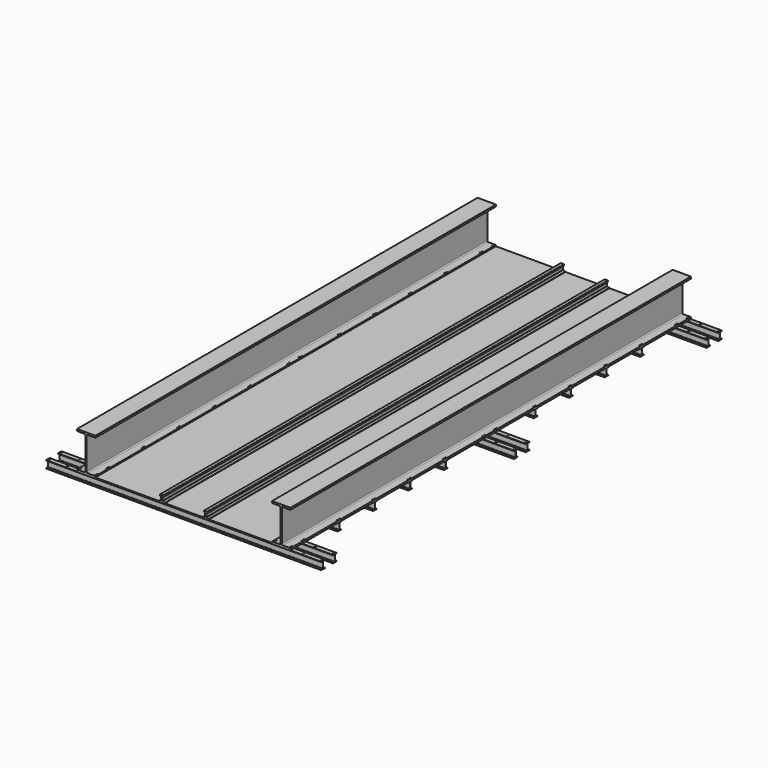
from build123d import *

# Parameters (mm, degrees)
F1_DEPTH      = 4250
F3_DEPTH      = 12
F5_DEPTH      = 4250
F5_DEPTH_BACK = 4250
F7_DEPTH      = 2336.4
F7_DEPTH_BACK = 2336.4
F8_DEPTH      = 1811.4
F8_DEPTH_BACK = 1811.4
F10_D         = 17
F10_DEPTH     = 35
F10_TIP       = 5.1073152617
F10_2_D       = 17
F10_2_DEPTH   = 35
F10_2_TIP     = 5.1073152617
F10_3_D       = 17
F10_3_DEPTH   = 35
F10_3_TIP     = 5.1073152617
F10_4_D       = 17
F10_4_DEPTH   = 35
F10_4_TIP     = 5.1073152617
F10_5_D       = 17
F10_5_DEPTH   = 35
F10_5_TIP     = 5.1073152617
F10_6_D       = 17
F10_6_DEPTH   = 35
F10_6_TIP     = 5.1073152617
F12_D         = 17
F12_DEPTH     = 50
F12_TIP       = 5.1073152617
F12_2_D       = 17
F12_2_DEPTH   = 50
F12_2_TIP     = 5.1073152617
F12_3_D       = 17
F12_3_DEPTH   = 50
F12_3_TIP     = 5.1073152617
F12_4_D       = 17
F12_4_DEPTH   = 50
F12_4_TIP     = 5.1073152617
F12_5_D       = 17
F12_5_DEPTH   = 50
F12_5_TIP     = 5.1073152617
F12_6_D       = 17
F12_6_DEPTH   = 50
F12_6_TIP     = 5.1073152617
F12_7_D       = 17
F12_7_DEPTH   = 50
F12_7_TIP     = 5.1073152617
F12_8_D       = 17
F12_8_DEPTH   = 50
F12_8_TIP     = 5.1073152617
F12_9_D       = 17
F12_9_DEPTH   = 50
F12_9_TIP     = 5.1073152617
F13_D         = 17
F13_DEPTH     = 50
F13_TIP       = 5.1073152617
F13_2_D       = 17
F13_2_DEPTH   = 50
F13_2_TIP     = 5.1073152617
F13_3_D       = 17
F13_3_DEPTH   = 50
F13_3_TIP     = 5.1073152617
F13_4_D       = 17
F13_4_DEPTH   = 50
F13_4_TIP     = 5.1073152617
F13_5_D       = 17
F13_5_DEPTH   = 50
F13_5_TIP     = 5.1073152617
F13_6_D       = 17
F13_6_DEPTH   = 50
F13_6_TIP     = 5.1073152617
F13_7_D       = 17
F13_7_DEPTH   = 50
F13_7_TIP     = 5.1073152617
F13_8_D       = 17
F13_8_DEPTH   = 50
F13_8_TIP     = 5.1073152617
F13_9_D       = 17
F13_9_DEPTH   = 50
F13_9_TIP     = 5.1073152617


# Not quite as in the source:
# - a feature names something its author has since deleted; it is built from what else it names


with BuildPart() as f1:
    # F0 (on Front) → F1 (new body, symmetric)
    with BuildSketch(Plane.XZ):
        with BuildLine():
            Line((-425.45, 0), (-320.68, 0))
            ThreePointArc((-320.68, 0), (-319.5557002179, 0.4657002179), (-319.09, 1.59))
            Line((-319.09, 1.59), (-319.09, 5.7241462765))
            ThreePointArc((-319.09, 5.7241462765), (-319.4356530306, 6.7139445487), (-320.3223278236, 7.2733946795))
            Line((-320.3223278236, 7.2733946795), (-355.8434391951, 15.4740894086))
            ThreePointArc((-355.8434391951, 15.4740894086), (-359.384561796, 17.7083713773), (-360.765, 21.66133932))
            Line((-360.765, 21.66133932), (-360.765, 74.78866068))
            ThreePointArc((-360.765, 74.78866068), (-359.384561796, 78.7416286227), (-355.8434391951, 80.9759105914))
            Line((-355.8434391951, 80.9759105914), (-344.1323278236, 83.6796336898))
            ThreePointArc((-344.1323278236, 83.6796336898), (-343.2456530306, 84.2390838206), (-342.9, 85.2288820928))
            Line((-342.9, 85.2288820928), (-342.9, 100.01))
            ThreePointArc((-342.9, 100.01), (-345.2255721574, 105.6244278426), (-350.84, 107.95))
            Line((-350.84, 107.95), (-373.065, 107.95))
            Line((-373.065, 107.95), (-395.29, 107.95))
            ThreePointArc((-395.29, 107.95), (-400.9044278426, 105.6244278426), (-403.23, 100.01))
            Line((-403.23, 100.01), (-403.23, 85.2288820928))
            ThreePointArc((-403.23, 85.2288820928), (-402.8843469694, 84.2390838206), (-401.9976721764, 83.6796336898))
            Line((-401.9976721764, 83.6796336898), (-390.2865608049, 80.9759105914))
            ThreePointArc((-390.2865608049, 80.9759105914), (-386.745438204, 78.7416286227), (-385.365, 74.78866068))
            Line((-385.365, 74.78866068), (-385.365, 21.66133932))
            ThreePointArc((-385.365, 21.66133932), (-386.745438204, 17.7083713773), (-390.2865608049, 15.4740894086))
            Line((-390.2865608049, 15.4740894086), (-425.8076721764, 7.2733946795))
            ThreePointArc((-425.8076721764, 7.2733946795), (-426.6943469694, 6.7139445487), (-427.04, 5.7241462765))
            Line((-427.04, 5.7241462765), (-427.04, 1.59))
            ThreePointArc((-427.04, 1.59), (-426.5742997821, 0.4657002179), (-425.45, 0))
        make_face()
    extrude(amount=F1_DEPTH, both=True)


with BuildPart() as f1b:
    # F0 (on Front) → F1, piece 2 (new body, symmetric)
    with BuildSketch(Plane.XZ):
        with BuildLine():
            ThreePointArc((350.84, 107.95), (345.2255721574, 105.6244278426), (342.9, 100.01))
            Line((342.9, 100.01), (342.9, 85.2288820928))
            ThreePointArc((342.9, 85.2288820928), (343.2456530306, 84.2390838206), (344.1323278236, 83.6796336898))
            Line((344.1323278236, 83.6796336898), (355.8434391951, 80.9759105914))
            ThreePointArc((355.8434391951, 80.9759105914), (359.384561796, 78.7416286227), (360.765, 74.78866068))
            Line((360.765, 74.78866068), (360.765, 21.66133932))
            ThreePointArc((360.765, 21.66133932), (359.384561796, 17.7083713773), (355.8434391951, 15.4740894086))
            Line((355.8434391951, 15.4740894086), (320.3223278236, 7.2733946795))
            ThreePointArc((320.3223278236, 7.2733946795), (319.4356530306, 6.7139445487), (319.09, 5.7241462765))
            Line((319.09, 5.7241462765), (319.09, 1.59))
            ThreePointArc((319.09, 1.59), (319.5557002179, 0.4657002179), (320.68, 0))
            Line((320.68, 0), (425.45, 0))
            ThreePointArc((425.45, 0), (426.5742997821, 0.4657002179), (427.04, 1.59))
            Line((427.04, 1.59), (427.04, 5.7241462765))
            ThreePointArc((427.04, 5.7241462765), (426.6943469694, 6.7139445487), (425.8076721764, 7.2733946795))
            Line((425.8076721764, 7.2733946795), (390.2865608049, 15.4740894086))
            ThreePointArc((390.2865608049, 15.4740894086), (386.745438204, 17.7083713773), (385.365, 21.66133932))
            Line((385.365, 21.66133932), (385.365, 74.78866068))
            ThreePointArc((385.365, 74.78866068), (386.745438204, 78.7416286227), (390.2865608049, 80.9759105914))
            Line((390.2865608049, 80.9759105914), (401.9976721764, 83.6796336898))
            ThreePointArc((401.9976721764, 83.6796336898), (402.8843469694, 84.2390838206), (403.23, 85.2288820928))
            Line((403.23, 85.2288820928), (403.23, 100.01))
            ThreePointArc((403.23, 100.01), (400.9044278426, 105.6244278426), (395.29, 107.95))
            Line((395.29, 107.95), (373.065, 107.95))
            Line((373.065, 107.95), (350.84, 107.95))
        make_face()
    extrude(amount=F1_DEPTH, both=True)


with BuildPart() as f3:
    # F2 (on Top) → F3 (new body)
    with BuildSketch(Plane.XY):
        Polygon((425.8076721764, 4250), (390.2865608049, 4250), (0, 4250), (-1500, 4250), (-1500, -4250), (0, -4250), (1500, -4250), (1500, 4250), align=None)
    extrude(amount=-F3_DEPTH)


with BuildPart() as f5:
    # F4 (on Front) → F5 (new body, two sides)
    with BuildSketch(Plane.XZ) as f5_sk:
        with BuildLine():
            Line((-1811.4, -12), (-1500, -12))
            Line((-1500, -12), (-1500, 19.4))
            Line((-1500, 19.4), (-1630, 19.4))
            ThreePointArc((-1630, 19.4), (-1641.6672618896, 24.2327381104), (-1646.5, 35.9))
            Line((-1646.5, 35.9), (-1646.5, 305.9))
            Line((-1646.5, 305.9), (-1646.5, 575.9))
            ThreePointArc((-1646.5, 575.9), (-1641.6672618896, 587.5672618896), (-1630, 592.4))
            Line((-1630, 592.4), (-1500, 592.4))
            Line((-1500, 592.4), (-1500, 623.8))
            Line((-1500, 623.8), (-1811.4, 623.8))
            Line((-1811.4, 623.8), (-1811.4, 592.4))
            Line((-1811.4, 592.4), (-1681.4, 592.4))
            ThreePointArc((-1681.4, 592.4), (-1669.7327381104, 587.5672618896), (-1664.9, 575.9))
            Line((-1664.9, 575.9), (-1664.9, 305.9))
            Line((-1664.9, 305.9), (-1664.9, 35.9))
            ThreePointArc((-1664.9, 35.9), (-1669.7327381104, 24.2327381104), (-1681.4, 19.4))
            Line((-1681.4, 19.4), (-1811.4, 19.4))
            Line((-1811.4, 19.4), (-1811.4, -12))
        make_face()
    extrude(amount=F5_DEPTH)
    extrude(f5_sk.sketch, amount=-F5_DEPTH_BACK)

    # F12 (one way)
    with BuildSketch(Plane.XY.offset(19.4)):
        with Locations((-1791.4, -4234), (1791.4, -4234), (1791.4, -4190), (-1791.4, -3984), (-1791.4, -3940), (-1791.4, -3231.8), (-1791.4, -3187.8), (-1520.9798002243, -3187.8), (-1520, -3231.8), (1791.4, -3231.8), (1520, -3231.8), (1520.9798002243, -3187.8), (1791.4, -3187.8), (1791.4, -3984), (1520.9798002243, -3984), (1520, -3940), (1791.4, -3940), (1520, -4234), (1520.9798002243, -4190), (-1520, -4233.9999999999), (-1520.9798002243, -4189.9999999999), (-1520.9798002243, -3984), (-1520, -3940), (-1791.4, -2479.6), (-1520, -2479.6), (-1520.9798002243, -2435.6), (-1791.4, -2435.6), (-1791.4, -1727.4), (-1791.4, -1683.4), (-1520.9798002243, -1683.4), (-1520, -1727.4), (-1791.4, -975.2), (-1791.4, -931.2), (-1520.9798002243, -931.2), (-1520, -975.2), (-1520.9798002243, -147), (-1791.4, -147), (-1791.4, -103), (-1520, -103), (1791.4, -103), (1520, -103), (1520.9798002243, -147), (1791.4, -147), (1520.9798002243, -931.2), (1791.4, -931.2), (1791.4, -975.2), (1520, -975.2), (1520.9798002243, -1683.4), (1520, -1727.4), (1791.4, -1727.4), (1791.4, -1683.4), (1520.9798002243, -2435.6), (1791.4, -2435.6), (1791.4, -2479.6), (1520, -2479.6), (-1791.4, -4190)):
            Circle(F12_D / 2)
    extrude(amount=-F12_DEPTH, mode=Mode.SUBTRACT)
    with Locations(Plane.XY.offset(19.4)):
        with Locations((-1791.4, -4234), (1791.4, -4234), (1791.4, -4190), (-1791.4, -3984), (-1791.4, -3940), (-1791.4, -3231.8), (-1791.4, -3187.8), (-1520.9798002243, -3187.8), (-1520, -3231.8), (1791.4, -3231.8), (1520, -3231.8), (1520.9798002243, -3187.8), (1791.4, -3187.8), (1791.4, -3984), (1520.9798002243, -3984), (1520, -3940), (1791.4, -3940), (1520, -4234), (1520.9798002243, -4190), (-1520, -4233.9999999999), (-1520.9798002243, -4189.9999999999), (-1520.9798002243, -3984), (-1520, -3940), (-1791.4, -2479.6), (-1520, -2479.6), (-1520.9798002243, -2435.6), (-1791.4, -2435.6), (-1791.4, -1727.4), (-1791.4, -1683.4), (-1520.9798002243, -1683.4), (-1520, -1727.4), (-1791.4, -975.2), (-1791.4, -931.2), (-1520.9798002243, -931.2), (-1520, -975.2), (-1520.9798002243, -147), (-1791.4, -147), (-1791.4, -103), (-1520, -103), (1791.4, -103), (1520, -103), (1520.9798002243, -147), (1791.4, -147), (1520.9798002243, -931.2), (1791.4, -931.2), (1791.4, -975.2), (1520, -975.2), (1520.9798002243, -1683.4), (1520, -1727.4), (1791.4, -1727.4), (1791.4, -1683.4), (1520.9798002243, -2435.6), (1791.4, -2435.6), (1791.4, -2479.6), (1520, -2479.6), (-1791.4, -4190)):
            with Locations((0, 0, -(F12_DEPTH + F12_TIP / 2))):  # 118° drill point
                Cone(0, F12_D / 2, F12_TIP, mode=Mode.SUBTRACT)

    # F13 (one way)
    with BuildSketch(Plane.XY.offset(19.4)):
        with Locations((1791.4, 931.2), (1520.9798002243, 931.2), (1520, 975.2), (1791.4, 975.2), (1791.4, 1683.4), (1520.9798002243, 1683.4), (1520, 1727.4), (1791.4, 1727.4), (1791.4, 2435.6), (1520.9798002243, 2435.6), (1520, 2479.6), (1791.4, 2479.6), (1520.9798002243, 3187.8), (1791.4, 3187.8), (1791.4, 3231.8), (1520, 3231.8), (1791.4, 3940), (1791.4, 3984), (1520.9798002243, 3984), (1520, 3940), (1791.4, 4190), (1520.9798002243, 4190), (1791.4, 4234), (1520, 4234), (-1520, 4233.9999999999), (-1520.9798002243, 4189.9999999999), (-1791.4, 4190), (-1791.4, 4234), (-1520.9798002243, 3984), (-1520, 3940), (-1791.4, 3940), (-1791.4, 3984), (-1520, 3231.8), (-1520.9798002243, 3187.8), (-1791.4, 3187.8), (-1791.4, 3231.8), (-1520, 2479.6), (-1520.9798002243, 2435.6), (-1791.4, 2435.6), (-1791.4, 2479.6), (-1520, 1727.4), (-1520.9798002243, 1683.4), (-1791.4, 1683.4), (-1791.4, 1727.4), (-1520, 975.2), (-1520.9798002243, 931.2), (-1791.4, 931.2), (-1791.4, 975.2), (-1791.4, 147), (-1520.9798002243, 147), (-1520, 103), (-1791.4, 103), (1791.4, 147), (1791.4, 103), (1520, 103), (1520.9798002243, 147)):
            Circle(F13_D / 2)
    extrude(amount=-F13_DEPTH, mode=Mode.SUBTRACT)
    with Locations(Plane.XY.offset(19.4)):
        with Locations((1791.4, 931.2), (1520.9798002243, 931.2), (1520, 975.2), (1791.4, 975.2), (1791.4, 1683.4), (1520.9798002243, 1683.4), (1520, 1727.4), (1791.4, 1727.4), (1791.4, 2435.6), (1520.9798002243, 2435.6), (1520, 2479.6), (1791.4, 2479.6), (1520.9798002243, 3187.8), (1791.4, 3187.8), (1791.4, 3231.8), (1520, 3231.8), (1791.4, 3940), (1791.4, 3984), (1520.9798002243, 3984), (1520, 3940), (1791.4, 4190), (1520.9798002243, 4190), (1791.4, 4234), (1520, 4234), (-1520, 4233.9999999999), (-1520.9798002243, 4189.9999999999), (-1791.4, 4190), (-1791.4, 4234), (-1520.9798002243, 3984), (-1520, 3940), (-1791.4, 3940), (-1791.4, 3984), (-1520, 3231.8), (-1520.9798002243, 3187.8), (-1791.4, 3187.8), (-1791.4, 3231.8), (-1520, 2479.6), (-1520.9798002243, 2435.6), (-1791.4, 2435.6), (-1791.4, 2479.6), (-1520, 1727.4), (-1520.9798002243, 1683.4), (-1791.4, 1683.4), (-1791.4, 1727.4), (-1520, 975.2), (-1520.9798002243, 931.2), (-1791.4, 931.2), (-1791.4, 975.2), (-1791.4, 147), (-1520.9798002243, 147), (-1520, 103), (-1791.4, 103), (1791.4, 147), (1791.4, 103), (1520, 103), (1520.9798002243, 147)):
            with Locations((0, 0, -(F13_DEPTH + F13_TIP / 2))):  # 118° drill point
                Cone(0, F13_D / 2, F13_TIP, mode=Mode.SUBTRACT)


with BuildPart() as f5b:
    # F4 (on Front) → F5, piece 2 (new body, two sides)
    with BuildSketch(Plane.XZ) as f5_2_sk:
        with BuildLine():
            Line((1811.4, 592.4), (1811.4, 623.8))
            Line((1811.4, 623.8), (1500, 623.8))
            Line((1500, 623.8), (1500, 592.4))
            Line((1500, 592.4), (1630, 592.4))
            ThreePointArc((1630, 592.4), (1641.6672618896, 587.5672618896), (1646.5, 575.9))
            Line((1646.5, 575.9), (1646.5, 305.9))
            Line((1646.5, 305.9), (1646.5, 35.9))
            ThreePointArc((1646.5, 35.9), (1641.6672618896, 24.2327381104), (1630, 19.4))
            Line((1630, 19.4), (1500, 19.4))
            Line((1500, 19.4), (1500, -12))
            Line((1500, -12), (1811.4, -12))
            Line((1811.4, -12), (1811.4, 19.4))
            Line((1811.4, 19.4), (1681.4, 19.4))
            ThreePointArc((1681.4, 19.4), (1669.7327381104, 24.2327381104), (1664.9, 35.9))
            Line((1664.9, 35.9), (1664.9, 305.9))
            Line((1664.9, 305.9), (1664.9, 575.9))
            ThreePointArc((1664.9, 575.9), (1669.7327381104, 587.5672618896), (1681.4, 592.4))
            Line((1681.4, 592.4), (1811.4, 592.4))
        make_face()
    extrude(amount=F5_DEPTH)
    extrude(f5_2_sk.sketch, amount=-F5_DEPTH_BACK)

    # F12#2 (one way)
    with BuildSketch(Plane.XY.offset(19.4)):
        with Locations((-1791.4, -4234), (1791.4, -4234), (1791.4, -4190), (-1791.4, -3984), (-1791.4, -3940), (-1791.4, -3231.8), (-1791.4, -3187.8), (-1520.9798002243, -3187.8), (-1520, -3231.8), (1791.4, -3231.8), (1520, -3231.8), (1520.9798002243, -3187.8), (1791.4, -3187.8), (1791.4, -3984), (1520.9798002243, -3984), (1520, -3940), (1791.4, -3940), (1520, -4234), (1520.9798002243, -4190), (-1520, -4233.9999999999), (-1520.9798002243, -4189.9999999999), (-1520.9798002243, -3984), (-1520, -3940), (-1791.4, -2479.6), (-1520, -2479.6), (-1520.9798002243, -2435.6), (-1791.4, -2435.6), (-1791.4, -1727.4), (-1791.4, -1683.4), (-1520.9798002243, -1683.4), (-1520, -1727.4), (-1791.4, -975.2), (-1791.4, -931.2), (-1520.9798002243, -931.2), (-1520, -975.2), (-1520.9798002243, -147), (-1791.4, -147), (-1791.4, -103), (-1520, -103), (1791.4, -103), (1520, -103), (1520.9798002243, -147), (1791.4, -147), (1520.9798002243, -931.2), (1791.4, -931.2), (1791.4, -975.2), (1520, -975.2), (1520.9798002243, -1683.4), (1520, -1727.4), (1791.4, -1727.4), (1791.4, -1683.4), (1520.9798002243, -2435.6), (1791.4, -2435.6), (1791.4, -2479.6), (1520, -2479.6), (-1791.4, -4190)):
            Circle(F12_2_D / 2)
    extrude(amount=-F12_2_DEPTH, mode=Mode.SUBTRACT)
    with Locations(Plane.XY.offset(19.4)):
        with Locations((-1791.4, -4234), (1791.4, -4234), (1791.4, -4190), (-1791.4, -3984), (-1791.4, -3940), (-1791.4, -3231.8), (-1791.4, -3187.8), (-1520.9798002243, -3187.8), (-1520, -3231.8), (1791.4, -3231.8), (1520, -3231.8), (1520.9798002243, -3187.8), (1791.4, -3187.8), (1791.4, -3984), (1520.9798002243, -3984), (1520, -3940), (1791.4, -3940), (1520, -4234), (1520.9798002243, -4190), (-1520, -4233.9999999999), (-1520.9798002243, -4189.9999999999), (-1520.9798002243, -3984), (-1520, -3940), (-1791.4, -2479.6), (-1520, -2479.6), (-1520.9798002243, -2435.6), (-1791.4, -2435.6), (-1791.4, -1727.4), (-1791.4, -1683.4), (-1520.9798002243, -1683.4), (-1520, -1727.4), (-1791.4, -975.2), (-1791.4, -931.2), (-1520.9798002243, -931.2), (-1520, -975.2), (-1520.9798002243, -147), (-1791.4, -147), (-1791.4, -103), (-1520, -103), (1791.4, -103), (1520, -103), (1520.9798002243, -147), (1791.4, -147), (1520.9798002243, -931.2), (1791.4, -931.2), (1791.4, -975.2), (1520, -975.2), (1520.9798002243, -1683.4), (1520, -1727.4), (1791.4, -1727.4), (1791.4, -1683.4), (1520.9798002243, -2435.6), (1791.4, -2435.6), (1791.4, -2479.6), (1520, -2479.6), (-1791.4, -4190)):
            with Locations((0, 0, -(F12_2_DEPTH + F12_2_TIP / 2))):  # 118° drill point
                Cone(0, F12_2_D / 2, F12_2_TIP, mode=Mode.SUBTRACT)

    # F13#2 (one way)
    with BuildSketch(Plane.XY.offset(19.4)):
        with Locations((1791.4, 931.2), (1520.9798002243, 931.2), (1520, 975.2), (1791.4, 975.2), (1791.4, 1683.4), (1520.9798002243, 1683.4), (1520, 1727.4), (1791.4, 1727.4), (1791.4, 2435.6), (1520.9798002243, 2435.6), (1520, 2479.6), (1791.4, 2479.6), (1520.9798002243, 3187.8), (1791.4, 3187.8), (1791.4, 3231.8), (1520, 3231.8), (1791.4, 3940), (1791.4, 3984), (1520.9798002243, 3984), (1520, 3940), (1791.4, 4190), (1520.9798002243, 4190), (1791.4, 4234), (1520, 4234), (-1520, 4233.9999999999), (-1520.9798002243, 4189.9999999999), (-1791.4, 4190), (-1791.4, 4234), (-1520.9798002243, 3984), (-1520, 3940), (-1791.4, 3940), (-1791.4, 3984), (-1520, 3231.8), (-1520.9798002243, 3187.8), (-1791.4, 3187.8), (-1791.4, 3231.8), (-1520, 2479.6), (-1520.9798002243, 2435.6), (-1791.4, 2435.6), (-1791.4, 2479.6), (-1520, 1727.4), (-1520.9798002243, 1683.4), (-1791.4, 1683.4), (-1791.4, 1727.4), (-1520, 975.2), (-1520.9798002243, 931.2), (-1791.4, 931.2), (-1791.4, 975.2), (-1791.4, 147), (-1520.9798002243, 147), (-1520, 103), (-1791.4, 103), (1791.4, 147), (1791.4, 103), (1520, 103), (1520.9798002243, 147)):
            Circle(F13_2_D / 2)
    extrude(amount=-F13_2_DEPTH, mode=Mode.SUBTRACT)
    with Locations(Plane.XY.offset(19.4)):
        with Locations((1791.4, 931.2), (1520.9798002243, 931.2), (1520, 975.2), (1791.4, 975.2), (1791.4, 1683.4), (1520.9798002243, 1683.4), (1520, 1727.4), (1791.4, 1727.4), (1791.4, 2435.6), (1520.9798002243, 2435.6), (1520, 2479.6), (1791.4, 2479.6), (1520.9798002243, 3187.8), (1791.4, 3187.8), (1791.4, 3231.8), (1520, 3231.8), (1791.4, 3940), (1791.4, 3984), (1520.9798002243, 3984), (1520, 3940), (1791.4, 4190), (1520.9798002243, 4190), (1791.4, 4234), (1520, 4234), (-1520, 4233.9999999999), (-1520.9798002243, 4189.9999999999), (-1791.4, 4190), (-1791.4, 4234), (-1520.9798002243, 3984), (-1520, 3940), (-1791.4, 3940), (-1791.4, 3984), (-1520, 3231.8), (-1520.9798002243, 3187.8), (-1791.4, 3187.8), (-1791.4, 3231.8), (-1520, 2479.6), (-1520.9798002243, 2435.6), (-1791.4, 2435.6), (-1791.4, 2479.6), (-1520, 1727.4), (-1520.9798002243, 1683.4), (-1791.4, 1683.4), (-1791.4, 1727.4), (-1520, 975.2), (-1520.9798002243, 931.2), (-1791.4, 931.2), (-1791.4, 975.2), (-1791.4, 147), (-1520.9798002243, 147), (-1520, 103), (-1791.4, 103), (1791.4, 147), (1791.4, 103), (1520, 103), (1520.9798002243, 147)):
            with Locations((0, 0, -(F13_2_DEPTH + F13_2_TIP / 2))):  # 118° drill point
                Cone(0, F13_2_D / 2, F13_2_TIP, mode=Mode.SUBTRACT)


with BuildPart() as f7:
    # F6 (on Right) → F7 (new body, two sides)
    with BuildSketch(Plane.YZ) as f7_sk:
        with BuildLine():
            Line((163, -12), (87, -12))
            Line((87, -12), (87, -19.6))
            Line((87, -19.6), (115.4, -19.6))
            ThreePointArc((115.4, -19.6), (120.774011537, -21.825988463), (123, -27.2))
            Line((123, -27.2), (123, -123.8))
            ThreePointArc((123, -123.8), (120.774011537, -129.174011537), (115.4, -131.4))
            Line((115.4, -131.4), (87, -131.4))
            Line((87, -131.4), (87, -139))
            Line((87, -139), (163, -139))
            Line((163, -139), (163, -131.4))
            Line((163, -131.4), (134.6, -131.4))
            ThreePointArc((134.6, -131.4), (129.225988463, -129.174011537), (127, -123.8))
            Line((127, -123.8), (127, -27.2))
            ThreePointArc((127, -27.2), (129.225988463, -21.825988463), (134.6, -19.6))
            Line((134.6, -19.6), (163, -19.6))
            Line((163, -19.6), (163, -12))
        make_face()
    extrude(amount=-F7_DEPTH)
    extrude(f7_sk.sketch, amount=F7_DEPTH_BACK)

    # F10
    with Locations(Plane.XY.offset(-12)):
        with Locations((-2312.4, 4190), (-2312.4, 4234), (-2004.4, 4190), (-2004.4, 4234), (-2004.4, 3984), (-2004.4, 3940), (-2312.4, 3940), (-2312.4, 3984), (2312.4, 3984), (2312.4, 3940), (2004.4, 3940), (2004.4, 3984), (2004.4, 4190), (2312.4, 4190), (2004.4, 4234), (2312.4, 4234), (2312.4, 103), (2004.4, 103), (2004.4, 147), (2312.4, 147), (2004.4, -103), (2312.4, -103), (2312.4, -147), (2004.4, -147), (-2312.4, 147), (-2004.4, 147), (-2004.4, 103), (-2312.4, 103), (-2312.4, -103), (-2004.4, -103), (-2004.4, -147), (-2312.4, -147), (2312.4, -3940), (2312.4, -3984), (2004.4, -3940), (2004.4, -3984), (2312.4, -4190), (2312.4, -4234), (2004.4, -4190), (2004.4, -4234), (-2004.4, -4190), (-2004.4, -4234), (-2312.4, -4234), (-2312.4, -4190), (-2312.4, -3984), (-2004.4, -3984), (-2004.4, -3940), (-2312.4, -3940)):
            Hole(F10_D / 2, depth=F10_DEPTH)
            with Locations((0, 0, -(F10_DEPTH + F10_TIP / 2))):  # 118° drill point
                Cone(0, F10_D / 2, F10_TIP, mode=Mode.SUBTRACT)

    # F13#3 (one way)
    with BuildSketch(Plane.XY.offset(19.4)):
        with Locations((1791.4, 931.2), (1520.9798002243, 931.2), (1520, 975.2), (1791.4, 975.2), (1791.4, 1683.4), (1520.9798002243, 1683.4), (1520, 1727.4), (1791.4, 1727.4), (1791.4, 2435.6), (1520.9798002243, 2435.6), (1520, 2479.6), (1791.4, 2479.6), (1520.9798002243, 3187.8), (1791.4, 3187.8), (1791.4, 3231.8), (1520, 3231.8), (1791.4, 3940), (1791.4, 3984), (1520.9798002243, 3984), (1520, 3940), (1791.4, 4190), (1520.9798002243, 4190), (1791.4, 4234), (1520, 4234), (-1520, 4233.9999999999), (-1520.9798002243, 4189.9999999999), (-1791.4, 4190), (-1791.4, 4234), (-1520.9798002243, 3984), (-1520, 3940), (-1791.4, 3940), (-1791.4, 3984), (-1520, 3231.8), (-1520.9798002243, 3187.8), (-1791.4, 3187.8), (-1791.4, 3231.8), (-1520, 2479.6), (-1520.9798002243, 2435.6), (-1791.4, 2435.6), (-1791.4, 2479.6), (-1520, 1727.4), (-1520.9798002243, 1683.4), (-1791.4, 1683.4), (-1791.4, 1727.4), (-1520, 975.2), (-1520.9798002243, 931.2), (-1791.4, 931.2), (-1791.4, 975.2), (-1791.4, 147), (-1520.9798002243, 147), (-1520, 103), (-1791.4, 103), (1791.4, 147), (1791.4, 103), (1520, 103), (1520.9798002243, 147)):
            Circle(F13_3_D / 2)
    extrude(amount=-F13_3_DEPTH, mode=Mode.SUBTRACT)
    with Locations(Plane.XY.offset(19.4)):
        with Locations((1791.4, 931.2), (1520.9798002243, 931.2), (1520, 975.2), (1791.4, 975.2), (1791.4, 1683.4), (1520.9798002243, 1683.4), (1520, 1727.4), (1791.4, 1727.4), (1791.4, 2435.6), (1520.9798002243, 2435.6), (1520, 2479.6), (1791.4, 2479.6), (1520.9798002243, 3187.8), (1791.4, 3187.8), (1791.4, 3231.8), (1520, 3231.8), (1791.4, 3940), (1791.4, 3984), (1520.9798002243, 3984), (1520, 3940), (1791.4, 4190), (1520.9798002243, 4190), (1791.4, 4234), (1520, 4234), (-1520, 4233.9999999999), (-1520.9798002243, 4189.9999999999), (-1791.4, 4190), (-1791.4, 4234), (-1520.9798002243, 3984), (-1520, 3940), (-1791.4, 3940), (-1791.4, 3984), (-1520, 3231.8), (-1520.9798002243, 3187.8), (-1791.4, 3187.8), (-1791.4, 3231.8), (-1520, 2479.6), (-1520.9798002243, 2435.6), (-1791.4, 2435.6), (-1791.4, 2479.6), (-1520, 1727.4), (-1520.9798002243, 1683.4), (-1791.4, 1683.4), (-1791.4, 1727.4), (-1520, 975.2), (-1520.9798002243, 931.2), (-1791.4, 931.2), (-1791.4, 975.2), (-1791.4, 147), (-1520.9798002243, 147), (-1520, 103), (-1791.4, 103), (1791.4, 147), (1791.4, 103), (1520, 103), (1520.9798002243, 147)):
            with Locations((0, 0, -(F13_3_DEPTH + F13_3_TIP / 2))):  # 118° drill point
                Cone(0, F13_3_D / 2, F13_3_TIP, mode=Mode.SUBTRACT)


with BuildPart() as f7b:
    # F6 (on Right) → F7, piece 2 (new body, two sides)
    with BuildSketch(Plane.YZ) as f7_2_sk:
        with BuildLine():
            Line((-87, -12), (-163, -12))
            Line((-163, -12), (-163, -19.6))
            Line((-163, -19.6), (-134.6, -19.6))
            ThreePointArc((-134.6, -19.6), (-129.225988463, -21.825988463), (-127, -27.2))
            Line((-127, -27.2), (-127, -123.8))
            ThreePointArc((-127, -123.8), (-129.225988463, -129.174011537), (-134.6, -131.4))
            Line((-134.6, -131.4), (-163, -131.4))
            Line((-163, -131.4), (-163, -139))
            Line((-163, -139), (-87, -139))
            Line((-87, -139), (-87, -131.4))
            Line((-87, -131.4), (-115.4, -131.4))
            ThreePointArc((-115.4, -131.4), (-120.774011537, -129.174011537), (-123, -123.8))
            Line((-123, -123.8), (-123, -27.2))
            ThreePointArc((-123, -27.2), (-120.774011537, -21.825988463), (-115.4, -19.6))
            Line((-115.4, -19.6), (-87, -19.6))
            Line((-87, -19.6), (-87, -12))
        make_face()
    extrude(amount=-F7_DEPTH)
    extrude(f7_2_sk.sketch, amount=F7_DEPTH_BACK)

    # F10#2
    with Locations(Plane.XY.offset(-12)):
        with Locations((-2312.4, 4190), (-2312.4, 4234), (-2004.4, 4190), (-2004.4, 4234), (-2004.4, 3984), (-2004.4, 3940), (-2312.4, 3940), (-2312.4, 3984), (2312.4, 3984), (2312.4, 3940), (2004.4, 3940), (2004.4, 3984), (2004.4, 4190), (2312.4, 4190), (2004.4, 4234), (2312.4, 4234), (2312.4, 103), (2004.4, 103), (2004.4, 147), (2312.4, 147), (2004.4, -103), (2312.4, -103), (2312.4, -147), (2004.4, -147), (-2312.4, 147), (-2004.4, 147), (-2004.4, 103), (-2312.4, 103), (-2312.4, -103), (-2004.4, -103), (-2004.4, -147), (-2312.4, -147), (2312.4, -3940), (2312.4, -3984), (2004.4, -3940), (2004.4, -3984), (2312.4, -4190), (2312.4, -4234), (2004.4, -4190), (2004.4, -4234), (-2004.4, -4190), (-2004.4, -4234), (-2312.4, -4234), (-2312.4, -4190), (-2312.4, -3984), (-2004.4, -3984), (-2004.4, -3940), (-2312.4, -3940)):
            Hole(F10_2_D / 2, depth=F10_2_DEPTH)
            with Locations((0, 0, -(F10_2_DEPTH + F10_2_TIP / 2))):  # 118° drill point
                Cone(0, F10_2_D / 2, F10_2_TIP, mode=Mode.SUBTRACT)

    # F12#3 (one way)
    with BuildSketch(Plane.XY.offset(19.4)):
        with Locations((-1791.4, -4234), (1791.4, -4234), (1791.4, -4190), (-1791.4, -3984), (-1791.4, -3940), (-1791.4, -3231.8), (-1791.4, -3187.8), (-1520.9798002243, -3187.8), (-1520, -3231.8), (1791.4, -3231.8), (1520, -3231.8), (1520.9798002243, -3187.8), (1791.4, -3187.8), (1791.4, -3984), (1520.9798002243, -3984), (1520, -3940), (1791.4, -3940), (1520, -4234), (1520.9798002243, -4190), (-1520, -4233.9999999999), (-1520.9798002243, -4189.9999999999), (-1520.9798002243, -3984), (-1520, -3940), (-1791.4, -2479.6), (-1520, -2479.6), (-1520.9798002243, -2435.6), (-1791.4, -2435.6), (-1791.4, -1727.4), (-1791.4, -1683.4), (-1520.9798002243, -1683.4), (-1520, -1727.4), (-1791.4, -975.2), (-1791.4, -931.2), (-1520.9798002243, -931.2), (-1520, -975.2), (-1520.9798002243, -147), (-1791.4, -147), (-1791.4, -103), (-1520, -103), (1791.4, -103), (1520, -103), (1520.9798002243, -147), (1791.4, -147), (1520.9798002243, -931.2), (1791.4, -931.2), (1791.4, -975.2), (1520, -975.2), (1520.9798002243, -1683.4), (1520, -1727.4), (1791.4, -1727.4), (1791.4, -1683.4), (1520.9798002243, -2435.6), (1791.4, -2435.6), (1791.4, -2479.6), (1520, -2479.6), (-1791.4, -4190)):
            Circle(F12_3_D / 2)
    extrude(amount=-F12_3_DEPTH, mode=Mode.SUBTRACT)
    with Locations(Plane.XY.offset(19.4)):
        with Locations((-1791.4, -4234), (1791.4, -4234), (1791.4, -4190), (-1791.4, -3984), (-1791.4, -3940), (-1791.4, -3231.8), (-1791.4, -3187.8), (-1520.9798002243, -3187.8), (-1520, -3231.8), (1791.4, -3231.8), (1520, -3231.8), (1520.9798002243, -3187.8), (1791.4, -3187.8), (1791.4, -3984), (1520.9798002243, -3984), (1520, -3940), (1791.4, -3940), (1520, -4234), (1520.9798002243, -4190), (-1520, -4233.9999999999), (-1520.9798002243, -4189.9999999999), (-1520.9798002243, -3984), (-1520, -3940), (-1791.4, -2479.6), (-1520, -2479.6), (-1520.9798002243, -2435.6), (-1791.4, -2435.6), (-1791.4, -1727.4), (-1791.4, -1683.4), (-1520.9798002243, -1683.4), (-1520, -1727.4), (-1791.4, -975.2), (-1791.4, -931.2), (-1520.9798002243, -931.2), (-1520, -975.2), (-1520.9798002243, -147), (-1791.4, -147), (-1791.4, -103), (-1520, -103), (1791.4, -103), (1520, -103), (1520.9798002243, -147), (1791.4, -147), (1520.9798002243, -931.2), (1791.4, -931.2), (1791.4, -975.2), (1520, -975.2), (1520.9798002243, -1683.4), (1520, -1727.4), (1791.4, -1727.4), (1791.4, -1683.4), (1520.9798002243, -2435.6), (1791.4, -2435.6), (1791.4, -2479.6), (1520, -2479.6), (-1791.4, -4190)):
            with Locations((0, 0, -(F12_3_DEPTH + F12_3_TIP / 2))):  # 118° drill point
                Cone(0, F12_3_D / 2, F12_3_TIP, mode=Mode.SUBTRACT)


with BuildPart() as f7c:
    # F6 (on Right) → F7, piece 3 (new body, two sides)
    with BuildSketch(Plane.YZ) as f7_3_sk:
        with BuildLine():
            Line((-4174, -12), (-4250, -12))
            Line((-4250, -12), (-4250, -19.6))
            Line((-4250, -19.6), (-4221.6, -19.6))
            ThreePointArc((-4221.6, -19.6), (-4216.225988463, -21.825988463), (-4214, -27.2))
            Line((-4214, -27.2), (-4214, -123.8))
            ThreePointArc((-4214, -123.8), (-4216.225988463, -129.174011537), (-4221.6, -131.4))
            Line((-4221.6, -131.4), (-4214, -131.4))
            Line((-4214, -131.4), (-4210, -131.4))
            Line((-4210, -131.4), (-4202.4, -131.4))
            ThreePointArc((-4202.4, -131.4), (-4207.774011537, -129.174011537), (-4210, -123.8))
            Line((-4210, -123.8), (-4210, -27.2))
            ThreePointArc((-4210, -27.2), (-4207.774011537, -21.825988463), (-4202.4, -19.6))
            Line((-4202.4, -19.6), (-4174, -19.6))
            Line((-4174, -19.6), (-4174, -12))
        make_face()
        Polygon((-4214, -131.4), (-4221.6, -131.4), (-4250, -131.4), (-4250, -139), (-4174, -139), (-4174, -131.4), (-4202.4, -131.4), (-4210, -131.4), align=None)
    extrude(amount=-F7_DEPTH)
    extrude(f7_3_sk.sketch, amount=F7_DEPTH_BACK)

    # F10#3
    with Locations(Plane.XY.offset(-12)):
        with Locations((-2312.4, 4190), (-2312.4, 4234), (-2004.4, 4190), (-2004.4, 4234), (-2004.4, 3984), (-2004.4, 3940), (-2312.4, 3940), (-2312.4, 3984), (2312.4, 3984), (2312.4, 3940), (2004.4, 3940), (2004.4, 3984), (2004.4, 4190), (2312.4, 4190), (2004.4, 4234), (2312.4, 4234), (2312.4, 103), (2004.4, 103), (2004.4, 147), (2312.4, 147), (2004.4, -103), (2312.4, -103), (2312.4, -147), (2004.4, -147), (-2312.4, 147), (-2004.4, 147), (-2004.4, 103), (-2312.4, 103), (-2312.4, -103), (-2004.4, -103), (-2004.4, -147), (-2312.4, -147), (2312.4, -3940), (2312.4, -3984), (2004.4, -3940), (2004.4, -3984), (2312.4, -4190), (2312.4, -4234), (2004.4, -4190), (2004.4, -4234), (-2004.4, -4190), (-2004.4, -4234), (-2312.4, -4234), (-2312.4, -4190), (-2312.4, -3984), (-2004.4, -3984), (-2004.4, -3940), (-2312.4, -3940)):
            Hole(F10_3_D / 2, depth=F10_3_DEPTH)
            with Locations((0, 0, -(F10_3_DEPTH + F10_3_TIP / 2))):  # 118° drill point
                Cone(0, F10_3_D / 2, F10_3_TIP, mode=Mode.SUBTRACT)

    # F12#4 (one way)
    with BuildSketch(Plane.XY.offset(19.4)):
        with Locations((-1791.4, -4234), (1791.4, -4234), (1791.4, -4190), (-1791.4, -3984), (-1791.4, -3940), (-1791.4, -3231.8), (-1791.4, -3187.8), (-1520.9798002243, -3187.8), (-1520, -3231.8), (1791.4, -3231.8), (1520, -3231.8), (1520.9798002243, -3187.8), (1791.4, -3187.8), (1791.4, -3984), (1520.9798002243, -3984), (1520, -3940), (1791.4, -3940), (1520, -4234), (1520.9798002243, -4190), (-1520, -4233.9999999999), (-1520.9798002243, -4189.9999999999), (-1520.9798002243, -3984), (-1520, -3940), (-1791.4, -2479.6), (-1520, -2479.6), (-1520.9798002243, -2435.6), (-1791.4, -2435.6), (-1791.4, -1727.4), (-1791.4, -1683.4), (-1520.9798002243, -1683.4), (-1520, -1727.4), (-1791.4, -975.2), (-1791.4, -931.2), (-1520.9798002243, -931.2), (-1520, -975.2), (-1520.9798002243, -147), (-1791.4, -147), (-1791.4, -103), (-1520, -103), (1791.4, -103), (1520, -103), (1520.9798002243, -147), (1791.4, -147), (1520.9798002243, -931.2), (1791.4, -931.2), (1791.4, -975.2), (1520, -975.2), (1520.9798002243, -1683.4), (1520, -1727.4), (1791.4, -1727.4), (1791.4, -1683.4), (1520.9798002243, -2435.6), (1791.4, -2435.6), (1791.4, -2479.6), (1520, -2479.6), (-1791.4, -4190)):
            Circle(F12_4_D / 2)
    extrude(amount=-F12_4_DEPTH, mode=Mode.SUBTRACT)
    with Locations(Plane.XY.offset(19.4)):
        with Locations((-1791.4, -4234), (1791.4, -4234), (1791.4, -4190), (-1791.4, -3984), (-1791.4, -3940), (-1791.4, -3231.8), (-1791.4, -3187.8), (-1520.9798002243, -3187.8), (-1520, -3231.8), (1791.4, -3231.8), (1520, -3231.8), (1520.9798002243, -3187.8), (1791.4, -3187.8), (1791.4, -3984), (1520.9798002243, -3984), (1520, -3940), (1791.4, -3940), (1520, -4234), (1520.9798002243, -4190), (-1520, -4233.9999999999), (-1520.9798002243, -4189.9999999999), (-1520.9798002243, -3984), (-1520, -3940), (-1791.4, -2479.6), (-1520, -2479.6), (-1520.9798002243, -2435.6), (-1791.4, -2435.6), (-1791.4, -1727.4), (-1791.4, -1683.4), (-1520.9798002243, -1683.4), (-1520, -1727.4), (-1791.4, -975.2), (-1791.4, -931.2), (-1520.9798002243, -931.2), (-1520, -975.2), (-1520.9798002243, -147), (-1791.4, -147), (-1791.4, -103), (-1520, -103), (1791.4, -103), (1520, -103), (1520.9798002243, -147), (1791.4, -147), (1520.9798002243, -931.2), (1791.4, -931.2), (1791.4, -975.2), (1520, -975.2), (1520.9798002243, -1683.4), (1520, -1727.4), (1791.4, -1727.4), (1791.4, -1683.4), (1520.9798002243, -2435.6), (1791.4, -2435.6), (1791.4, -2479.6), (1520, -2479.6), (-1791.4, -4190)):
            with Locations((0, 0, -(F12_4_DEPTH + F12_4_TIP / 2))):  # 118° drill point
                Cone(0, F12_4_D / 2, F12_4_TIP, mode=Mode.SUBTRACT)


with BuildPart() as f7d:
    # F6 (on Right) → F7, piece 4 (new body, two sides)
    with BuildSketch(Plane.YZ) as f7_4_sk:
        with BuildLine():
            Line((-3924, -12), (-4000, -12))
            Line((-4000, -12), (-4000, -19.6))
            Line((-4000, -19.6), (-3971.6, -19.6))
            ThreePointArc((-3971.6, -19.6), (-3966.225988463, -21.825988463), (-3964, -27.2))
            Line((-3964, -27.2), (-3964, -123.8))
            ThreePointArc((-3964, -123.8), (-3966.225988463, -129.174011537), (-3971.6, -131.4))
            Line((-3971.6, -131.4), (-4000, -131.4))
            Line((-4000, -131.4), (-4000, -139))
            Line((-4000, -139), (-3924, -139))
            Line((-3924, -139), (-3924, -131.4))
            Line((-3924, -131.4), (-3952.4, -131.4))
            ThreePointArc((-3952.4, -131.4), (-3957.774011537, -129.174011537), (-3960, -123.8))
            Line((-3960, -123.8), (-3960, -27.2))
            ThreePointArc((-3960, -27.2), (-3957.774011537, -21.825988463), (-3952.4, -19.6))
            Line((-3952.4, -19.6), (-3924, -19.6))
            Line((-3924, -19.6), (-3924, -12))
        make_face()
    extrude(amount=-F7_DEPTH)
    extrude(f7_4_sk.sketch, amount=F7_DEPTH_BACK)

    # F10#4
    with Locations(Plane.XY.offset(-12)):
        with Locations((-2312.4, 4190), (-2312.4, 4234), (-2004.4, 4190), (-2004.4, 4234), (-2004.4, 3984), (-2004.4, 3940), (-2312.4, 3940), (-2312.4, 3984), (2312.4, 3984), (2312.4, 3940), (2004.4, 3940), (2004.4, 3984), (2004.4, 4190), (2312.4, 4190), (2004.4, 4234), (2312.4, 4234), (2312.4, 103), (2004.4, 103), (2004.4, 147), (2312.4, 147), (2004.4, -103), (2312.4, -103), (2312.4, -147), (2004.4, -147), (-2312.4, 147), (-2004.4, 147), (-2004.4, 103), (-2312.4, 103), (-2312.4, -103), (-2004.4, -103), (-2004.4, -147), (-2312.4, -147), (2312.4, -3940), (2312.4, -3984), (2004.4, -3940), (2004.4, -3984), (2312.4, -4190), (2312.4, -4234), (2004.4, -4190), (2004.4, -4234), (-2004.4, -4190), (-2004.4, -4234), (-2312.4, -4234), (-2312.4, -4190), (-2312.4, -3984), (-2004.4, -3984), (-2004.4, -3940), (-2312.4, -3940)):
            Hole(F10_4_D / 2, depth=F10_4_DEPTH)
            with Locations((0, 0, -(F10_4_DEPTH + F10_4_TIP / 2))):  # 118° drill point
                Cone(0, F10_4_D / 2, F10_4_TIP, mode=Mode.SUBTRACT)

    # F12#5 (one way)
    with BuildSketch(Plane.XY.offset(19.4)):
        with Locations((-1791.4, -4234), (1791.4, -4234), (1791.4, -4190), (-1791.4, -3984), (-1791.4, -3940), (-1791.4, -3231.8), (-1791.4, -3187.8), (-1520.9798002243, -3187.8), (-1520, -3231.8), (1791.4, -3231.8), (1520, -3231.8), (1520.9798002243, -3187.8), (1791.4, -3187.8), (1791.4, -3984), (1520.9798002243, -3984), (1520, -3940), (1791.4, -3940), (1520, -4234), (1520.9798002243, -4190), (-1520, -4233.9999999999), (-1520.9798002243, -4189.9999999999), (-1520.9798002243, -3984), (-1520, -3940), (-1791.4, -2479.6), (-1520, -2479.6), (-1520.9798002243, -2435.6), (-1791.4, -2435.6), (-1791.4, -1727.4), (-1791.4, -1683.4), (-1520.9798002243, -1683.4), (-1520, -1727.4), (-1791.4, -975.2), (-1791.4, -931.2), (-1520.9798002243, -931.2), (-1520, -975.2), (-1520.9798002243, -147), (-1791.4, -147), (-1791.4, -103), (-1520, -103), (1791.4, -103), (1520, -103), (1520.9798002243, -147), (1791.4, -147), (1520.9798002243, -931.2), (1791.4, -931.2), (1791.4, -975.2), (1520, -975.2), (1520.9798002243, -1683.4), (1520, -1727.4), (1791.4, -1727.4), (1791.4, -1683.4), (1520.9798002243, -2435.6), (1791.4, -2435.6), (1791.4, -2479.6), (1520, -2479.6), (-1791.4, -4190)):
            Circle(F12_5_D / 2)
    extrude(amount=-F12_5_DEPTH, mode=Mode.SUBTRACT)
    with Locations(Plane.XY.offset(19.4)):
        with Locations((-1791.4, -4234), (1791.4, -4234), (1791.4, -4190), (-1791.4, -3984), (-1791.4, -3940), (-1791.4, -3231.8), (-1791.4, -3187.8), (-1520.9798002243, -3187.8), (-1520, -3231.8), (1791.4, -3231.8), (1520, -3231.8), (1520.9798002243, -3187.8), (1791.4, -3187.8), (1791.4, -3984), (1520.9798002243, -3984), (1520, -3940), (1791.4, -3940), (1520, -4234), (1520.9798002243, -4190), (-1520, -4233.9999999999), (-1520.9798002243, -4189.9999999999), (-1520.9798002243, -3984), (-1520, -3940), (-1791.4, -2479.6), (-1520, -2479.6), (-1520.9798002243, -2435.6), (-1791.4, -2435.6), (-1791.4, -1727.4), (-1791.4, -1683.4), (-1520.9798002243, -1683.4), (-1520, -1727.4), (-1791.4, -975.2), (-1791.4, -931.2), (-1520.9798002243, -931.2), (-1520, -975.2), (-1520.9798002243, -147), (-1791.4, -147), (-1791.4, -103), (-1520, -103), (1791.4, -103), (1520, -103), (1520.9798002243, -147), (1791.4, -147), (1520.9798002243, -931.2), (1791.4, -931.2), (1791.4, -975.2), (1520, -975.2), (1520.9798002243, -1683.4), (1520, -1727.4), (1791.4, -1727.4), (1791.4, -1683.4), (1520.9798002243, -2435.6), (1791.4, -2435.6), (1791.4, -2479.6), (1520, -2479.6), (-1791.4, -4190)):
            with Locations((0, 0, -(F12_5_DEPTH + F12_5_TIP / 2))):  # 118° drill point
                Cone(0, F12_5_D / 2, F12_5_TIP, mode=Mode.SUBTRACT)


with BuildPart() as f7e:
    # F6 (on Right) → F7, piece 5 (new body, two sides)
    with BuildSketch(Plane.YZ) as f7_5_sk:
        with BuildLine():
            Line((4250, -12), (4174, -12))
            Line((4174, -12), (4174, -19.6))
            Line((4174, -19.6), (4202.4, -19.6))
            ThreePointArc((4202.4, -19.6), (4207.774011537, -21.825988463), (4210, -27.2))
            Line((4210, -27.2), (4210, -123.8))
            ThreePointArc((4210, -123.8), (4207.774011537, -129.174011537), (4202.4, -131.4))
            Line((4202.4, -131.4), (4174, -131.4))
            Line((4174, -131.4), (4174, -139))
            Line((4174, -139), (4250, -139))
            Line((4250, -139), (4250, -131.4))
            Line((4250, -131.4), (4221.6, -131.4))
            ThreePointArc((4221.6, -131.4), (4216.225988463, -129.174011537), (4214, -123.8))
            Line((4214, -123.8), (4214, -27.2))
            ThreePointArc((4214, -27.2), (4216.225988463, -21.825988463), (4221.6, -19.6))
            Line((4221.6, -19.6), (4250, -19.6))
            Line((4250, -19.6), (4250, -12))
        make_face()
    extrude(amount=-F7_DEPTH)
    extrude(f7_5_sk.sketch, amount=F7_DEPTH_BACK)

    # F10#5
    with Locations(Plane.XY.offset(-12)):
        with Locations((-2312.4, 4190), (-2312.4, 4234), (-2004.4, 4190), (-2004.4, 4234), (-2004.4, 3984), (-2004.4, 3940), (-2312.4, 3940), (-2312.4, 3984), (2312.4, 3984), (2312.4, 3940), (2004.4, 3940), (2004.4, 3984), (2004.4, 4190), (2312.4, 4190), (2004.4, 4234), (2312.4, 4234), (2312.4, 103), (2004.4, 103), (2004.4, 147), (2312.4, 147), (2004.4, -103), (2312.4, -103), (2312.4, -147), (2004.4, -147), (-2312.4, 147), (-2004.4, 147), (-2004.4, 103), (-2312.4, 103), (-2312.4, -103), (-2004.4, -103), (-2004.4, -147), (-2312.4, -147), (2312.4, -3940), (2312.4, -3984), (2004.4, -3940), (2004.4, -3984), (2312.4, -4190), (2312.4, -4234), (2004.4, -4190), (2004.4, -4234), (-2004.4, -4190), (-2004.4, -4234), (-2312.4, -4234), (-2312.4, -4190), (-2312.4, -3984), (-2004.4, -3984), (-2004.4, -3940), (-2312.4, -3940)):
            Hole(F10_5_D / 2, depth=F10_5_DEPTH)
            with Locations((0, 0, -(F10_5_DEPTH + F10_5_TIP / 2))):  # 118° drill point
                Cone(0, F10_5_D / 2, F10_5_TIP, mode=Mode.SUBTRACT)

    # F13#4 (one way)
    with BuildSketch(Plane.XY.offset(19.4)):
        with Locations((1791.4, 931.2), (1520.9798002243, 931.2), (1520, 975.2), (1791.4, 975.2), (1791.4, 1683.4), (1520.9798002243, 1683.4), (1520, 1727.4), (1791.4, 1727.4), (1791.4, 2435.6), (1520.9798002243, 2435.6), (1520, 2479.6), (1791.4, 2479.6), (1520.9798002243, 3187.8), (1791.4, 3187.8), (1791.4, 3231.8), (1520, 3231.8), (1791.4, 3940), (1791.4, 3984), (1520.9798002243, 3984), (1520, 3940), (1791.4, 4190), (1520.9798002243, 4190), (1791.4, 4234), (1520, 4234), (-1520, 4233.9999999999), (-1520.9798002243, 4189.9999999999), (-1791.4, 4190), (-1791.4, 4234), (-1520.9798002243, 3984), (-1520, 3940), (-1791.4, 3940), (-1791.4, 3984), (-1520, 3231.8), (-1520.9798002243, 3187.8), (-1791.4, 3187.8), (-1791.4, 3231.8), (-1520, 2479.6), (-1520.9798002243, 2435.6), (-1791.4, 2435.6), (-1791.4, 2479.6), (-1520, 1727.4), (-1520.9798002243, 1683.4), (-1791.4, 1683.4), (-1791.4, 1727.4), (-1520, 975.2), (-1520.9798002243, 931.2), (-1791.4, 931.2), (-1791.4, 975.2), (-1791.4, 147), (-1520.9798002243, 147), (-1520, 103), (-1791.4, 103), (1791.4, 147), (1791.4, 103), (1520, 103), (1520.9798002243, 147)):
            Circle(F13_4_D / 2)
    extrude(amount=-F13_4_DEPTH, mode=Mode.SUBTRACT)
    with Locations(Plane.XY.offset(19.4)):
        with Locations((1791.4, 931.2), (1520.9798002243, 931.2), (1520, 975.2), (1791.4, 975.2), (1791.4, 1683.4), (1520.9798002243, 1683.4), (1520, 1727.4), (1791.4, 1727.4), (1791.4, 2435.6), (1520.9798002243, 2435.6), (1520, 2479.6), (1791.4, 2479.6), (1520.9798002243, 3187.8), (1791.4, 3187.8), (1791.4, 3231.8), (1520, 3231.8), (1791.4, 3940), (1791.4, 3984), (1520.9798002243, 3984), (1520, 3940), (1791.4, 4190), (1520.9798002243, 4190), (1791.4, 4234), (1520, 4234), (-1520, 4233.9999999999), (-1520.9798002243, 4189.9999999999), (-1791.4, 4190), (-1791.4, 4234), (-1520.9798002243, 3984), (-1520, 3940), (-1791.4, 3940), (-1791.4, 3984), (-1520, 3231.8), (-1520.9798002243, 3187.8), (-1791.4, 3187.8), (-1791.4, 3231.8), (-1520, 2479.6), (-1520.9798002243, 2435.6), (-1791.4, 2435.6), (-1791.4, 2479.6), (-1520, 1727.4), (-1520.9798002243, 1683.4), (-1791.4, 1683.4), (-1791.4, 1727.4), (-1520, 975.2), (-1520.9798002243, 931.2), (-1791.4, 931.2), (-1791.4, 975.2), (-1791.4, 147), (-1520.9798002243, 147), (-1520, 103), (-1791.4, 103), (1791.4, 147), (1791.4, 103), (1520, 103), (1520.9798002243, 147)):
            with Locations((0, 0, -(F13_4_DEPTH + F13_4_TIP / 2))):  # 118° drill point
                Cone(0, F13_4_D / 2, F13_4_TIP, mode=Mode.SUBTRACT)


with BuildPart() as f7f:
    # F6 (on Right) → F7, piece 6 (new body, two sides)
    with BuildSketch(Plane.YZ) as f7_6_sk:
        with BuildLine():
            Line((4000, -12), (3924, -12))
            Line((3924, -12), (3924, -19.6))
            Line((3924, -19.6), (3952.4, -19.6))
            ThreePointArc((3952.4, -19.6), (3957.774011537, -21.825988463), (3960, -27.2))
            Line((3960, -27.2), (3960, -123.8))
            ThreePointArc((3960, -123.8), (3957.774011537, -129.174011537), (3952.4, -131.4))
            Line((3952.4, -131.4), (3924, -131.4))
            Line((3924, -131.4), (3924, -139))
            Line((3924, -139), (4000, -139))
            Line((4000, -139), (4000, -131.4))
            Line((4000, -131.4), (3971.6, -131.4))
            ThreePointArc((3971.6, -131.4), (3966.225988463, -129.174011537), (3964, -123.8))
            Line((3964, -123.8), (3964, -27.2))
            ThreePointArc((3964, -27.2), (3966.225988463, -21.825988463), (3971.6, -19.6))
            Line((3971.6, -19.6), (4000, -19.6))
            Line((4000, -19.6), (4000, -12))
        make_face()
    extrude(amount=-F7_DEPTH)
    extrude(f7_6_sk.sketch, amount=F7_DEPTH_BACK)

    # F10#6
    with Locations(Plane.XY.offset(-12)):
        with Locations((-2312.4, 4190), (-2312.4, 4234), (-2004.4, 4190), (-2004.4, 4234), (-2004.4, 3984), (-2004.4, 3940), (-2312.4, 3940), (-2312.4, 3984), (2312.4, 3984), (2312.4, 3940), (2004.4, 3940), (2004.4, 3984), (2004.4, 4190), (2312.4, 4190), (2004.4, 4234), (2312.4, 4234), (2312.4, 103), (2004.4, 103), (2004.4, 147), (2312.4, 147), (2004.4, -103), (2312.4, -103), (2312.4, -147), (2004.4, -147), (-2312.4, 147), (-2004.4, 147), (-2004.4, 103), (-2312.4, 103), (-2312.4, -103), (-2004.4, -103), (-2004.4, -147), (-2312.4, -147), (2312.4, -3940), (2312.4, -3984), (2004.4, -3940), (2004.4, -3984), (2312.4, -4190), (2312.4, -4234), (2004.4, -4190), (2004.4, -4234), (-2004.4, -4190), (-2004.4, -4234), (-2312.4, -4234), (-2312.4, -4190), (-2312.4, -3984), (-2004.4, -3984), (-2004.4, -3940), (-2312.4, -3940)):
            Hole(F10_6_D / 2, depth=F10_6_DEPTH)
            with Locations((0, 0, -(F10_6_DEPTH + F10_6_TIP / 2))):  # 118° drill point
                Cone(0, F10_6_D / 2, F10_6_TIP, mode=Mode.SUBTRACT)

    # F13#5 (one way)
    with BuildSketch(Plane.XY.offset(19.4)):
        with Locations((1791.4, 931.2), (1520.9798002243, 931.2), (1520, 975.2), (1791.4, 975.2), (1791.4, 1683.4), (1520.9798002243, 1683.4), (1520, 1727.4), (1791.4, 1727.4), (1791.4, 2435.6), (1520.9798002243, 2435.6), (1520, 2479.6), (1791.4, 2479.6), (1520.9798002243, 3187.8), (1791.4, 3187.8), (1791.4, 3231.8), (1520, 3231.8), (1791.4, 3940), (1791.4, 3984), (1520.9798002243, 3984), (1520, 3940), (1791.4, 4190), (1520.9798002243, 4190), (1791.4, 4234), (1520, 4234), (-1520, 4233.9999999999), (-1520.9798002243, 4189.9999999999), (-1791.4, 4190), (-1791.4, 4234), (-1520.9798002243, 3984), (-1520, 3940), (-1791.4, 3940), (-1791.4, 3984), (-1520, 3231.8), (-1520.9798002243, 3187.8), (-1791.4, 3187.8), (-1791.4, 3231.8), (-1520, 2479.6), (-1520.9798002243, 2435.6), (-1791.4, 2435.6), (-1791.4, 2479.6), (-1520, 1727.4), (-1520.9798002243, 1683.4), (-1791.4, 1683.4), (-1791.4, 1727.4), (-1520, 975.2), (-1520.9798002243, 931.2), (-1791.4, 931.2), (-1791.4, 975.2), (-1791.4, 147), (-1520.9798002243, 147), (-1520, 103), (-1791.4, 103), (1791.4, 147), (1791.4, 103), (1520, 103), (1520.9798002243, 147)):
            Circle(F13_5_D / 2)
    extrude(amount=-F13_5_DEPTH, mode=Mode.SUBTRACT)
    with Locations(Plane.XY.offset(19.4)):
        with Locations((1791.4, 931.2), (1520.9798002243, 931.2), (1520, 975.2), (1791.4, 975.2), (1791.4, 1683.4), (1520.9798002243, 1683.4), (1520, 1727.4), (1791.4, 1727.4), (1791.4, 2435.6), (1520.9798002243, 2435.6), (1520, 2479.6), (1791.4, 2479.6), (1520.9798002243, 3187.8), (1791.4, 3187.8), (1791.4, 3231.8), (1520, 3231.8), (1791.4, 3940), (1791.4, 3984), (1520.9798002243, 3984), (1520, 3940), (1791.4, 4190), (1520.9798002243, 4190), (1791.4, 4234), (1520, 4234), (-1520, 4233.9999999999), (-1520.9798002243, 4189.9999999999), (-1791.4, 4190), (-1791.4, 4234), (-1520.9798002243, 3984), (-1520, 3940), (-1791.4, 3940), (-1791.4, 3984), (-1520, 3231.8), (-1520.9798002243, 3187.8), (-1791.4, 3187.8), (-1791.4, 3231.8), (-1520, 2479.6), (-1520.9798002243, 2435.6), (-1791.4, 2435.6), (-1791.4, 2479.6), (-1520, 1727.4), (-1520.9798002243, 1683.4), (-1791.4, 1683.4), (-1791.4, 1727.4), (-1520, 975.2), (-1520.9798002243, 931.2), (-1791.4, 931.2), (-1791.4, 975.2), (-1791.4, 147), (-1520.9798002243, 147), (-1520, 103), (-1791.4, 103), (1791.4, 147), (1791.4, 103), (1520, 103), (1520.9798002243, 147)):
            with Locations((0, 0, -(F13_5_DEPTH + F13_5_TIP / 2))):  # 118° drill point
                Cone(0, F13_5_D / 2, F13_5_TIP, mode=Mode.SUBTRACT)


with BuildPart() as f8:
    # F6 (on Right) → F8 (new body, two sides)
    with BuildSketch(Plane.YZ) as f8_sk:
        with BuildLine():
            Line((-3171.8, -12), (-3247.8, -12))
            Line((-3247.8, -12), (-3247.8, -19.6))
            Line((-3247.8, -19.6), (-3219.4, -19.6))
            ThreePointArc((-3219.4, -19.6), (-3214.025988463, -21.825988463), (-3211.8, -27.2))
            Line((-3211.8, -27.2), (-3211.8, -123.8))
            ThreePointArc((-3211.8, -123.8), (-3214.025988463, -129.174011537), (-3219.4, -131.4))
            Line((-3219.4, -131.4), (-3247.8, -131.4))
            Line((-3247.8, -131.4), (-3247.8, -139))
            Line((-3247.8, -139), (-3171.8, -139))
            Line((-3171.8, -139), (-3171.8, -131.4))
            Line((-3171.8, -131.4), (-3200.2, -131.4))
            ThreePointArc((-3200.2, -131.4), (-3205.574011537, -129.174011537), (-3207.8, -123.8))
            Line((-3207.8, -123.8), (-3207.8, -27.2))
            ThreePointArc((-3207.8, -27.2), (-3205.574011537, -21.825988463), (-3200.2, -19.6))
            Line((-3200.2, -19.6), (-3171.8, -19.6))
            Line((-3171.8, -19.6), (-3171.8, -12))
        make_face()
    extrude(amount=-F8_DEPTH)
    extrude(f8_sk.sketch, amount=F8_DEPTH_BACK)

    # F12#6 (one way)
    with BuildSketch(Plane.XY.offset(19.4)):
        with Locations((-1791.4, -4234), (1791.4, -4234), (1791.4, -4190), (-1791.4, -3984), (-1791.4, -3940), (-1791.4, -3231.8), (-1791.4, -3187.8), (-1520.9798002243, -3187.8), (-1520, -3231.8), (1791.4, -3231.8), (1520, -3231.8), (1520.9798002243, -3187.8), (1791.4, -3187.8), (1791.4, -3984), (1520.9798002243, -3984), (1520, -3940), (1791.4, -3940), (1520, -4234), (1520.9798002243, -4190), (-1520, -4233.9999999999), (-1520.9798002243, -4189.9999999999), (-1520.9798002243, -3984), (-1520, -3940), (-1791.4, -2479.6), (-1520, -2479.6), (-1520.9798002243, -2435.6), (-1791.4, -2435.6), (-1791.4, -1727.4), (-1791.4, -1683.4), (-1520.9798002243, -1683.4), (-1520, -1727.4), (-1791.4, -975.2), (-1791.4, -931.2), (-1520.9798002243, -931.2), (-1520, -975.2), (-1520.9798002243, -147), (-1791.4, -147), (-1791.4, -103), (-1520, -103), (1791.4, -103), (1520, -103), (1520.9798002243, -147), (1791.4, -147), (1520.9798002243, -931.2), (1791.4, -931.2), (1791.4, -975.2), (1520, -975.2), (1520.9798002243, -1683.4), (1520, -1727.4), (1791.4, -1727.4), (1791.4, -1683.4), (1520.9798002243, -2435.6), (1791.4, -2435.6), (1791.4, -2479.6), (1520, -2479.6), (-1791.4, -4190)):
            Circle(F12_6_D / 2)
    extrude(amount=-F12_6_DEPTH, mode=Mode.SUBTRACT)
    with Locations(Plane.XY.offset(19.4)):
        with Locations((-1791.4, -4234), (1791.4, -4234), (1791.4, -4190), (-1791.4, -3984), (-1791.4, -3940), (-1791.4, -3231.8), (-1791.4, -3187.8), (-1520.9798002243, -3187.8), (-1520, -3231.8), (1791.4, -3231.8), (1520, -3231.8), (1520.9798002243, -3187.8), (1791.4, -3187.8), (1791.4, -3984), (1520.9798002243, -3984), (1520, -3940), (1791.4, -3940), (1520, -4234), (1520.9798002243, -4190), (-1520, -4233.9999999999), (-1520.9798002243, -4189.9999999999), (-1520.9798002243, -3984), (-1520, -3940), (-1791.4, -2479.6), (-1520, -2479.6), (-1520.9798002243, -2435.6), (-1791.4, -2435.6), (-1791.4, -1727.4), (-1791.4, -1683.4), (-1520.9798002243, -1683.4), (-1520, -1727.4), (-1791.4, -975.2), (-1791.4, -931.2), (-1520.9798002243, -931.2), (-1520, -975.2), (-1520.9798002243, -147), (-1791.4, -147), (-1791.4, -103), (-1520, -103), (1791.4, -103), (1520, -103), (1520.9798002243, -147), (1791.4, -147), (1520.9798002243, -931.2), (1791.4, -931.2), (1791.4, -975.2), (1520, -975.2), (1520.9798002243, -1683.4), (1520, -1727.4), (1791.4, -1727.4), (1791.4, -1683.4), (1520.9798002243, -2435.6), (1791.4, -2435.6), (1791.4, -2479.6), (1520, -2479.6), (-1791.4, -4190)):
            with Locations((0, 0, -(F12_6_DEPTH + F12_6_TIP / 2))):  # 118° drill point
                Cone(0, F12_6_D / 2, F12_6_TIP, mode=Mode.SUBTRACT)


with BuildPart() as f8b:
    # F6 (on Right) → F8, piece 2 (new body, two sides)
    with BuildSketch(Plane.YZ) as f8_2_sk:
        with BuildLine():
            Line((-2419.6, -12), (-2495.6, -12))
            Line((-2495.6, -12), (-2495.6, -19.6))
            Line((-2495.6, -19.6), (-2467.2, -19.6))
            ThreePointArc((-2467.2, -19.6), (-2461.825988463, -21.825988463), (-2459.6, -27.2))
            Line((-2459.6, -27.2), (-2459.6, -123.8))
            ThreePointArc((-2459.6, -123.8), (-2461.825988463, -129.174011537), (-2467.2, -131.4))
            Line((-2467.2, -131.4), (-2495.6, -131.4))
            Line((-2495.6, -131.4), (-2495.6, -139))
            Line((-2495.6, -139), (-2419.6, -139))
            Line((-2419.6, -139), (-2419.6, -131.4))
            Line((-2419.6, -131.4), (-2448, -131.4))
            ThreePointArc((-2448, -131.4), (-2453.374011537, -129.174011537), (-2455.6, -123.8))
            Line((-2455.6, -123.8), (-2455.6, -27.2))
            ThreePointArc((-2455.6, -27.2), (-2453.374011537, -21.825988463), (-2448, -19.6))
            Line((-2448, -19.6), (-2419.6, -19.6))
            Line((-2419.6, -19.6), (-2419.6, -12))
        make_face()
    extrude(amount=-F8_DEPTH)
    extrude(f8_2_sk.sketch, amount=F8_DEPTH_BACK)

    # F12#7 (one way)
    with BuildSketch(Plane.XY.offset(19.4)):
        with Locations((-1791.4, -4234), (1791.4, -4234), (1791.4, -4190), (-1791.4, -3984), (-1791.4, -3940), (-1791.4, -3231.8), (-1791.4, -3187.8), (-1520.9798002243, -3187.8), (-1520, -3231.8), (1791.4, -3231.8), (1520, -3231.8), (1520.9798002243, -3187.8), (1791.4, -3187.8), (1791.4, -3984), (1520.9798002243, -3984), (1520, -3940), (1791.4, -3940), (1520, -4234), (1520.9798002243, -4190), (-1520, -4233.9999999999), (-1520.9798002243, -4189.9999999999), (-1520.9798002243, -3984), (-1520, -3940), (-1791.4, -2479.6), (-1520, -2479.6), (-1520.9798002243, -2435.6), (-1791.4, -2435.6), (-1791.4, -1727.4), (-1791.4, -1683.4), (-1520.9798002243, -1683.4), (-1520, -1727.4), (-1791.4, -975.2), (-1791.4, -931.2), (-1520.9798002243, -931.2), (-1520, -975.2), (-1520.9798002243, -147), (-1791.4, -147), (-1791.4, -103), (-1520, -103), (1791.4, -103), (1520, -103), (1520.9798002243, -147), (1791.4, -147), (1520.9798002243, -931.2), (1791.4, -931.2), (1791.4, -975.2), (1520, -975.2), (1520.9798002243, -1683.4), (1520, -1727.4), (1791.4, -1727.4), (1791.4, -1683.4), (1520.9798002243, -2435.6), (1791.4, -2435.6), (1791.4, -2479.6), (1520, -2479.6), (-1791.4, -4190)):
            Circle(F12_7_D / 2)
    extrude(amount=-F12_7_DEPTH, mode=Mode.SUBTRACT)
    with Locations(Plane.XY.offset(19.4)):
        with Locations((-1791.4, -4234), (1791.4, -4234), (1791.4, -4190), (-1791.4, -3984), (-1791.4, -3940), (-1791.4, -3231.8), (-1791.4, -3187.8), (-1520.9798002243, -3187.8), (-1520, -3231.8), (1791.4, -3231.8), (1520, -3231.8), (1520.9798002243, -3187.8), (1791.4, -3187.8), (1791.4, -3984), (1520.9798002243, -3984), (1520, -3940), (1791.4, -3940), (1520, -4234), (1520.9798002243, -4190), (-1520, -4233.9999999999), (-1520.9798002243, -4189.9999999999), (-1520.9798002243, -3984), (-1520, -3940), (-1791.4, -2479.6), (-1520, -2479.6), (-1520.9798002243, -2435.6), (-1791.4, -2435.6), (-1791.4, -1727.4), (-1791.4, -1683.4), (-1520.9798002243, -1683.4), (-1520, -1727.4), (-1791.4, -975.2), (-1791.4, -931.2), (-1520.9798002243, -931.2), (-1520, -975.2), (-1520.9798002243, -147), (-1791.4, -147), (-1791.4, -103), (-1520, -103), (1791.4, -103), (1520, -103), (1520.9798002243, -147), (1791.4, -147), (1520.9798002243, -931.2), (1791.4, -931.2), (1791.4, -975.2), (1520, -975.2), (1520.9798002243, -1683.4), (1520, -1727.4), (1791.4, -1727.4), (1791.4, -1683.4), (1520.9798002243, -2435.6), (1791.4, -2435.6), (1791.4, -2479.6), (1520, -2479.6), (-1791.4, -4190)):
            with Locations((0, 0, -(F12_7_DEPTH + F12_7_TIP / 2))):  # 118° drill point
                Cone(0, F12_7_D / 2, F12_7_TIP, mode=Mode.SUBTRACT)


with BuildPart() as f8c:
    # F6 (on Right) → F8, piece 3 (new body, two sides)
    with BuildSketch(Plane.YZ) as f8_3_sk:
        with BuildLine():
            Line((-1667.4, -12), (-1743.4, -12))
            Line((-1743.4, -12), (-1743.4, -19.6))
            Line((-1743.4, -19.6), (-1715, -19.6))
            ThreePointArc((-1715, -19.6), (-1709.625988463, -21.825988463), (-1707.4, -27.2))
            Line((-1707.4, -27.2), (-1707.4, -123.8))
            ThreePointArc((-1707.4, -123.8), (-1709.625988463, -129.174011537), (-1715, -131.4))
            Line((-1715, -131.4), (-1743.4, -131.4))
            Line((-1743.4, -131.4), (-1743.4, -139))
            Line((-1743.4, -139), (-1667.4, -139))
            Line((-1667.4, -139), (-1667.4, -131.4))
            Line((-1667.4, -131.4), (-1695.8, -131.4))
            ThreePointArc((-1695.8, -131.4), (-1701.174011537, -129.174011537), (-1703.4, -123.8))
            Line((-1703.4, -123.8), (-1703.4, -27.2))
            ThreePointArc((-1703.4, -27.2), (-1701.174011537, -21.825988463), (-1695.8, -19.6))
            Line((-1695.8, -19.6), (-1667.4, -19.6))
            Line((-1667.4, -19.6), (-1667.4, -12))
        make_face()
    extrude(amount=-F8_DEPTH)
    extrude(f8_3_sk.sketch, amount=F8_DEPTH_BACK)

    # F12#8 (one way)
    with BuildSketch(Plane.XY.offset(19.4)):
        with Locations((-1791.4, -4234), (1791.4, -4234), (1791.4, -4190), (-1791.4, -3984), (-1791.4, -3940), (-1791.4, -3231.8), (-1791.4, -3187.8), (-1520.9798002243, -3187.8), (-1520, -3231.8), (1791.4, -3231.8), (1520, -3231.8), (1520.9798002243, -3187.8), (1791.4, -3187.8), (1791.4, -3984), (1520.9798002243, -3984), (1520, -3940), (1791.4, -3940), (1520, -4234), (1520.9798002243, -4190), (-1520, -4233.9999999999), (-1520.9798002243, -4189.9999999999), (-1520.9798002243, -3984), (-1520, -3940), (-1791.4, -2479.6), (-1520, -2479.6), (-1520.9798002243, -2435.6), (-1791.4, -2435.6), (-1791.4, -1727.4), (-1791.4, -1683.4), (-1520.9798002243, -1683.4), (-1520, -1727.4), (-1791.4, -975.2), (-1791.4, -931.2), (-1520.9798002243, -931.2), (-1520, -975.2), (-1520.9798002243, -147), (-1791.4, -147), (-1791.4, -103), (-1520, -103), (1791.4, -103), (1520, -103), (1520.9798002243, -147), (1791.4, -147), (1520.9798002243, -931.2), (1791.4, -931.2), (1791.4, -975.2), (1520, -975.2), (1520.9798002243, -1683.4), (1520, -1727.4), (1791.4, -1727.4), (1791.4, -1683.4), (1520.9798002243, -2435.6), (1791.4, -2435.6), (1791.4, -2479.6), (1520, -2479.6), (-1791.4, -4190)):
            Circle(F12_8_D / 2)
    extrude(amount=-F12_8_DEPTH, mode=Mode.SUBTRACT)
    with Locations(Plane.XY.offset(19.4)):
        with Locations((-1791.4, -4234), (1791.4, -4234), (1791.4, -4190), (-1791.4, -3984), (-1791.4, -3940), (-1791.4, -3231.8), (-1791.4, -3187.8), (-1520.9798002243, -3187.8), (-1520, -3231.8), (1791.4, -3231.8), (1520, -3231.8), (1520.9798002243, -3187.8), (1791.4, -3187.8), (1791.4, -3984), (1520.9798002243, -3984), (1520, -3940), (1791.4, -3940), (1520, -4234), (1520.9798002243, -4190), (-1520, -4233.9999999999), (-1520.9798002243, -4189.9999999999), (-1520.9798002243, -3984), (-1520, -3940), (-1791.4, -2479.6), (-1520, -2479.6), (-1520.9798002243, -2435.6), (-1791.4, -2435.6), (-1791.4, -1727.4), (-1791.4, -1683.4), (-1520.9798002243, -1683.4), (-1520, -1727.4), (-1791.4, -975.2), (-1791.4, -931.2), (-1520.9798002243, -931.2), (-1520, -975.2), (-1520.9798002243, -147), (-1791.4, -147), (-1791.4, -103), (-1520, -103), (1791.4, -103), (1520, -103), (1520.9798002243, -147), (1791.4, -147), (1520.9798002243, -931.2), (1791.4, -931.2), (1791.4, -975.2), (1520, -975.2), (1520.9798002243, -1683.4), (1520, -1727.4), (1791.4, -1727.4), (1791.4, -1683.4), (1520.9798002243, -2435.6), (1791.4, -2435.6), (1791.4, -2479.6), (1520, -2479.6), (-1791.4, -4190)):
            with Locations((0, 0, -(F12_8_DEPTH + F12_8_TIP / 2))):  # 118° drill point
                Cone(0, F12_8_D / 2, F12_8_TIP, mode=Mode.SUBTRACT)


with BuildPart() as f8d:
    # F6 (on Right) → F8, piece 4 (new body, two sides)
    with BuildSketch(Plane.YZ) as f8_4_sk:
        with BuildLine():
            Line((-915.2, -12), (-991.2, -12))
            Line((-991.2, -12), (-991.2, -19.6))
            Line((-991.2, -19.6), (-962.8, -19.6))
            ThreePointArc((-962.8, -19.6), (-957.425988463, -21.825988463), (-955.2, -27.2))
            Line((-955.2, -27.2), (-955.2, -123.8))
            ThreePointArc((-955.2, -123.8), (-957.425988463, -129.174011537), (-962.8, -131.4))
            Line((-962.8, -131.4), (-991.2, -131.4))
            Line((-991.2, -131.4), (-991.2, -139))
            Line((-991.2, -139), (-915.2, -139))
            Line((-915.2, -139), (-915.2, -131.4))
            Line((-915.2, -131.4), (-943.6, -131.4))
            ThreePointArc((-943.6, -131.4), (-948.974011537, -129.174011537), (-951.2, -123.8))
            Line((-951.2, -123.8), (-951.2, -27.2))
            ThreePointArc((-951.2, -27.2), (-948.974011537, -21.825988463), (-943.6, -19.6))
            Line((-943.6, -19.6), (-915.2, -19.6))
            Line((-915.2, -19.6), (-915.2, -12))
        make_face()
    extrude(amount=-F8_DEPTH)
    extrude(f8_4_sk.sketch, amount=F8_DEPTH_BACK)

    # F12#9 (one way)
    with BuildSketch(Plane.XY.offset(19.4)):
        with Locations((-1791.4, -4234), (1791.4, -4234), (1791.4, -4190), (-1791.4, -3984), (-1791.4, -3940), (-1791.4, -3231.8), (-1791.4, -3187.8), (-1520.9798002243, -3187.8), (-1520, -3231.8), (1791.4, -3231.8), (1520, -3231.8), (1520.9798002243, -3187.8), (1791.4, -3187.8), (1791.4, -3984), (1520.9798002243, -3984), (1520, -3940), (1791.4, -3940), (1520, -4234), (1520.9798002243, -4190), (-1520, -4233.9999999999), (-1520.9798002243, -4189.9999999999), (-1520.9798002243, -3984), (-1520, -3940), (-1791.4, -2479.6), (-1520, -2479.6), (-1520.9798002243, -2435.6), (-1791.4, -2435.6), (-1791.4, -1727.4), (-1791.4, -1683.4), (-1520.9798002243, -1683.4), (-1520, -1727.4), (-1791.4, -975.2), (-1791.4, -931.2), (-1520.9798002243, -931.2), (-1520, -975.2), (-1520.9798002243, -147), (-1791.4, -147), (-1791.4, -103), (-1520, -103), (1791.4, -103), (1520, -103), (1520.9798002243, -147), (1791.4, -147), (1520.9798002243, -931.2), (1791.4, -931.2), (1791.4, -975.2), (1520, -975.2), (1520.9798002243, -1683.4), (1520, -1727.4), (1791.4, -1727.4), (1791.4, -1683.4), (1520.9798002243, -2435.6), (1791.4, -2435.6), (1791.4, -2479.6), (1520, -2479.6), (-1791.4, -4190)):
            Circle(F12_9_D / 2)
    extrude(amount=-F12_9_DEPTH, mode=Mode.SUBTRACT)
    with Locations(Plane.XY.offset(19.4)):
        with Locations((-1791.4, -4234), (1791.4, -4234), (1791.4, -4190), (-1791.4, -3984), (-1791.4, -3940), (-1791.4, -3231.8), (-1791.4, -3187.8), (-1520.9798002243, -3187.8), (-1520, -3231.8), (1791.4, -3231.8), (1520, -3231.8), (1520.9798002243, -3187.8), (1791.4, -3187.8), (1791.4, -3984), (1520.9798002243, -3984), (1520, -3940), (1791.4, -3940), (1520, -4234), (1520.9798002243, -4190), (-1520, -4233.9999999999), (-1520.9798002243, -4189.9999999999), (-1520.9798002243, -3984), (-1520, -3940), (-1791.4, -2479.6), (-1520, -2479.6), (-1520.9798002243, -2435.6), (-1791.4, -2435.6), (-1791.4, -1727.4), (-1791.4, -1683.4), (-1520.9798002243, -1683.4), (-1520, -1727.4), (-1791.4, -975.2), (-1791.4, -931.2), (-1520.9798002243, -931.2), (-1520, -975.2), (-1520.9798002243, -147), (-1791.4, -147), (-1791.4, -103), (-1520, -103), (1791.4, -103), (1520, -103), (1520.9798002243, -147), (1791.4, -147), (1520.9798002243, -931.2), (1791.4, -931.2), (1791.4, -975.2), (1520, -975.2), (1520.9798002243, -1683.4), (1520, -1727.4), (1791.4, -1727.4), (1791.4, -1683.4), (1520.9798002243, -2435.6), (1791.4, -2435.6), (1791.4, -2479.6), (1520, -2479.6), (-1791.4, -4190)):
            with Locations((0, 0, -(F12_9_DEPTH + F12_9_TIP / 2))):  # 118° drill point
                Cone(0, F12_9_D / 2, F12_9_TIP, mode=Mode.SUBTRACT)


with BuildPart() as f8e:
    # F6 (on Right) → F8, piece 5 (new body, two sides)
    with BuildSketch(Plane.YZ) as f8_5_sk:
        with BuildLine():
            Line((991.2, -12), (915.2, -12))
            Line((915.2, -12), (915.2, -19.6))
            Line((915.2, -19.6), (943.6, -19.6))
            ThreePointArc((943.6, -19.6), (948.974011537, -21.825988463), (951.2, -27.2))
            Line((951.2, -27.2), (951.2, -123.8))
            ThreePointArc((951.2, -123.8), (948.974011537, -129.174011537), (943.6, -131.4))
            Line((943.6, -131.4), (915.2, -131.4))
            Line((915.2, -131.4), (915.2, -139))
            Line((915.2, -139), (991.2, -139))
            Line((991.2, -139), (991.2, -131.4))
            Line((991.2, -131.4), (962.8, -131.4))
            ThreePointArc((962.8, -131.4), (957.425988463, -129.174011537), (955.2, -123.8))
            Line((955.2, -123.8), (955.2, -27.2))
            ThreePointArc((955.2, -27.2), (957.425988463, -21.825988463), (962.8, -19.6))
            Line((962.8, -19.6), (991.2, -19.6))
            Line((991.2, -19.6), (991.2, -12))
        make_face()
    extrude(amount=-F8_DEPTH)
    extrude(f8_5_sk.sketch, amount=F8_DEPTH_BACK)

    # F13#6 (one way)
    with BuildSketch(Plane.XY.offset(19.4)):
        with Locations((1791.4, 931.2), (1520.9798002243, 931.2), (1520, 975.2), (1791.4, 975.2), (1791.4, 1683.4), (1520.9798002243, 1683.4), (1520, 1727.4), (1791.4, 1727.4), (1791.4, 2435.6), (1520.9798002243, 2435.6), (1520, 2479.6), (1791.4, 2479.6), (1520.9798002243, 3187.8), (1791.4, 3187.8), (1791.4, 3231.8), (1520, 3231.8), (1791.4, 3940), (1791.4, 3984), (1520.9798002243, 3984), (1520, 3940), (1791.4, 4190), (1520.9798002243, 4190), (1791.4, 4234), (1520, 4234), (-1520, 4233.9999999999), (-1520.9798002243, 4189.9999999999), (-1791.4, 4190), (-1791.4, 4234), (-1520.9798002243, 3984), (-1520, 3940), (-1791.4, 3940), (-1791.4, 3984), (-1520, 3231.8), (-1520.9798002243, 3187.8), (-1791.4, 3187.8), (-1791.4, 3231.8), (-1520, 2479.6), (-1520.9798002243, 2435.6), (-1791.4, 2435.6), (-1791.4, 2479.6), (-1520, 1727.4), (-1520.9798002243, 1683.4), (-1791.4, 1683.4), (-1791.4, 1727.4), (-1520, 975.2), (-1520.9798002243, 931.2), (-1791.4, 931.2), (-1791.4, 975.2), (-1791.4, 147), (-1520.9798002243, 147), (-1520, 103), (-1791.4, 103), (1791.4, 147), (1791.4, 103), (1520, 103), (1520.9798002243, 147)):
            Circle(F13_6_D / 2)
    extrude(amount=-F13_6_DEPTH, mode=Mode.SUBTRACT)
    with Locations(Plane.XY.offset(19.4)):
        with Locations((1791.4, 931.2), (1520.9798002243, 931.2), (1520, 975.2), (1791.4, 975.2), (1791.4, 1683.4), (1520.9798002243, 1683.4), (1520, 1727.4), (1791.4, 1727.4), (1791.4, 2435.6), (1520.9798002243, 2435.6), (1520, 2479.6), (1791.4, 2479.6), (1520.9798002243, 3187.8), (1791.4, 3187.8), (1791.4, 3231.8), (1520, 3231.8), (1791.4, 3940), (1791.4, 3984), (1520.9798002243, 3984), (1520, 3940), (1791.4, 4190), (1520.9798002243, 4190), (1791.4, 4234), (1520, 4234), (-1520, 4233.9999999999), (-1520.9798002243, 4189.9999999999), (-1791.4, 4190), (-1791.4, 4234), (-1520.9798002243, 3984), (-1520, 3940), (-1791.4, 3940), (-1791.4, 3984), (-1520, 3231.8), (-1520.9798002243, 3187.8), (-1791.4, 3187.8), (-1791.4, 3231.8), (-1520, 2479.6), (-1520.9798002243, 2435.6), (-1791.4, 2435.6), (-1791.4, 2479.6), (-1520, 1727.4), (-1520.9798002243, 1683.4), (-1791.4, 1683.4), (-1791.4, 1727.4), (-1520, 975.2), (-1520.9798002243, 931.2), (-1791.4, 931.2), (-1791.4, 975.2), (-1791.4, 147), (-1520.9798002243, 147), (-1520, 103), (-1791.4, 103), (1791.4, 147), (1791.4, 103), (1520, 103), (1520.9798002243, 147)):
            with Locations((0, 0, -(F13_6_DEPTH + F13_6_TIP / 2))):  # 118° drill point
                Cone(0, F13_6_D / 2, F13_6_TIP, mode=Mode.SUBTRACT)


with BuildPart() as f8f:
    # F6 (on Right) → F8, piece 6 (new body, two sides)
    with BuildSketch(Plane.YZ) as f8_6_sk:
        with BuildLine():
            Line((1743.4, -12), (1667.4, -12))
            Line((1667.4, -12), (1667.4, -19.6))
            Line((1667.4, -19.6), (1695.8, -19.6))
            ThreePointArc((1695.8, -19.6), (1701.174011537, -21.825988463), (1703.4, -27.2))
            Line((1703.4, -27.2), (1703.4, -123.8))
            ThreePointArc((1703.4, -123.8), (1701.174011537, -129.174011537), (1695.8, -131.4))
            Line((1695.8, -131.4), (1667.4, -131.4))
            Line((1667.4, -131.4), (1667.4, -139))
            Line((1667.4, -139), (1743.4, -139))
            Line((1743.4, -139), (1743.4, -131.4))
            Line((1743.4, -131.4), (1715, -131.4))
            ThreePointArc((1715, -131.4), (1709.625988463, -129.174011537), (1707.4, -123.8))
            Line((1707.4, -123.8), (1707.4, -27.2))
            ThreePointArc((1707.4, -27.2), (1709.625988463, -21.825988463), (1715, -19.6))
            Line((1715, -19.6), (1743.4, -19.6))
            Line((1743.4, -19.6), (1743.4, -12))
        make_face()
    extrude(amount=-F8_DEPTH)
    extrude(f8_6_sk.sketch, amount=F8_DEPTH_BACK)

    # F13#7 (one way)
    with BuildSketch(Plane.XY.offset(19.4)):
        with Locations((1791.4, 931.2), (1520.9798002243, 931.2), (1520, 975.2), (1791.4, 975.2), (1791.4, 1683.4), (1520.9798002243, 1683.4), (1520, 1727.4), (1791.4, 1727.4), (1791.4, 2435.6), (1520.9798002243, 2435.6), (1520, 2479.6), (1791.4, 2479.6), (1520.9798002243, 3187.8), (1791.4, 3187.8), (1791.4, 3231.8), (1520, 3231.8), (1791.4, 3940), (1791.4, 3984), (1520.9798002243, 3984), (1520, 3940), (1791.4, 4190), (1520.9798002243, 4190), (1791.4, 4234), (1520, 4234), (-1520, 4233.9999999999), (-1520.9798002243, 4189.9999999999), (-1791.4, 4190), (-1791.4, 4234), (-1520.9798002243, 3984), (-1520, 3940), (-1791.4, 3940), (-1791.4, 3984), (-1520, 3231.8), (-1520.9798002243, 3187.8), (-1791.4, 3187.8), (-1791.4, 3231.8), (-1520, 2479.6), (-1520.9798002243, 2435.6), (-1791.4, 2435.6), (-1791.4, 2479.6), (-1520, 1727.4), (-1520.9798002243, 1683.4), (-1791.4, 1683.4), (-1791.4, 1727.4), (-1520, 975.2), (-1520.9798002243, 931.2), (-1791.4, 931.2), (-1791.4, 975.2), (-1791.4, 147), (-1520.9798002243, 147), (-1520, 103), (-1791.4, 103), (1791.4, 147), (1791.4, 103), (1520, 103), (1520.9798002243, 147)):
            Circle(F13_7_D / 2)
    extrude(amount=-F13_7_DEPTH, mode=Mode.SUBTRACT)
    with Locations(Plane.XY.offset(19.4)):
        with Locations((1791.4, 931.2), (1520.9798002243, 931.2), (1520, 975.2), (1791.4, 975.2), (1791.4, 1683.4), (1520.9798002243, 1683.4), (1520, 1727.4), (1791.4, 1727.4), (1791.4, 2435.6), (1520.9798002243, 2435.6), (1520, 2479.6), (1791.4, 2479.6), (1520.9798002243, 3187.8), (1791.4, 3187.8), (1791.4, 3231.8), (1520, 3231.8), (1791.4, 3940), (1791.4, 3984), (1520.9798002243, 3984), (1520, 3940), (1791.4, 4190), (1520.9798002243, 4190), (1791.4, 4234), (1520, 4234), (-1520, 4233.9999999999), (-1520.9798002243, 4189.9999999999), (-1791.4, 4190), (-1791.4, 4234), (-1520.9798002243, 3984), (-1520, 3940), (-1791.4, 3940), (-1791.4, 3984), (-1520, 3231.8), (-1520.9798002243, 3187.8), (-1791.4, 3187.8), (-1791.4, 3231.8), (-1520, 2479.6), (-1520.9798002243, 2435.6), (-1791.4, 2435.6), (-1791.4, 2479.6), (-1520, 1727.4), (-1520.9798002243, 1683.4), (-1791.4, 1683.4), (-1791.4, 1727.4), (-1520, 975.2), (-1520.9798002243, 931.2), (-1791.4, 931.2), (-1791.4, 975.2), (-1791.4, 147), (-1520.9798002243, 147), (-1520, 103), (-1791.4, 103), (1791.4, 147), (1791.4, 103), (1520, 103), (1520.9798002243, 147)):
            with Locations((0, 0, -(F13_7_DEPTH + F13_7_TIP / 2))):  # 118° drill point
                Cone(0, F13_7_D / 2, F13_7_TIP, mode=Mode.SUBTRACT)


with BuildPart() as f8g:
    # F6 (on Right) → F8, piece 7 (new body, two sides)
    with BuildSketch(Plane.YZ) as f8_7_sk:
        with BuildLine():
            Line((2495.6, -12), (2419.6, -12))
            Line((2419.6, -12), (2419.6, -19.6))
            Line((2419.6, -19.6), (2448, -19.6))
            ThreePointArc((2448, -19.6), (2453.374011537, -21.825988463), (2455.6, -27.2))
            Line((2455.6, -27.2), (2455.6, -123.8))
            ThreePointArc((2455.6, -123.8), (2453.374011537, -129.174011537), (2448, -131.4))
            Line((2448, -131.4), (2419.6, -131.4))
            Line((2419.6, -131.4), (2419.6, -139))
            Line((2419.6, -139), (2495.6, -139))
            Line((2495.6, -139), (2495.6, -131.4))
            Line((2495.6, -131.4), (2467.2, -131.4))
            ThreePointArc((2467.2, -131.4), (2461.825988463, -129.174011537), (2459.6, -123.8))
            Line((2459.6, -123.8), (2459.6, -27.2))
            ThreePointArc((2459.6, -27.2), (2461.825988463, -21.825988463), (2467.2, -19.6))
            Line((2467.2, -19.6), (2495.6, -19.6))
            Line((2495.6, -19.6), (2495.6, -12))
        make_face()
    extrude(amount=-F8_DEPTH)
    extrude(f8_7_sk.sketch, amount=F8_DEPTH_BACK)

    # F13#8 (one way)
    with BuildSketch(Plane.XY.offset(19.4)):
        with Locations((1791.4, 931.2), (1520.9798002243, 931.2), (1520, 975.2), (1791.4, 975.2), (1791.4, 1683.4), (1520.9798002243, 1683.4), (1520, 1727.4), (1791.4, 1727.4), (1791.4, 2435.6), (1520.9798002243, 2435.6), (1520, 2479.6), (1791.4, 2479.6), (1520.9798002243, 3187.8), (1791.4, 3187.8), (1791.4, 3231.8), (1520, 3231.8), (1791.4, 3940), (1791.4, 3984), (1520.9798002243, 3984), (1520, 3940), (1791.4, 4190), (1520.9798002243, 4190), (1791.4, 4234), (1520, 4234), (-1520, 4233.9999999999), (-1520.9798002243, 4189.9999999999), (-1791.4, 4190), (-1791.4, 4234), (-1520.9798002243, 3984), (-1520, 3940), (-1791.4, 3940), (-1791.4, 3984), (-1520, 3231.8), (-1520.9798002243, 3187.8), (-1791.4, 3187.8), (-1791.4, 3231.8), (-1520, 2479.6), (-1520.9798002243, 2435.6), (-1791.4, 2435.6), (-1791.4, 2479.6), (-1520, 1727.4), (-1520.9798002243, 1683.4), (-1791.4, 1683.4), (-1791.4, 1727.4), (-1520, 975.2), (-1520.9798002243, 931.2), (-1791.4, 931.2), (-1791.4, 975.2), (-1791.4, 147), (-1520.9798002243, 147), (-1520, 103), (-1791.4, 103), (1791.4, 147), (1791.4, 103), (1520, 103), (1520.9798002243, 147)):
            Circle(F13_8_D / 2)
    extrude(amount=-F13_8_DEPTH, mode=Mode.SUBTRACT)
    with Locations(Plane.XY.offset(19.4)):
        with Locations((1791.4, 931.2), (1520.9798002243, 931.2), (1520, 975.2), (1791.4, 975.2), (1791.4, 1683.4), (1520.9798002243, 1683.4), (1520, 1727.4), (1791.4, 1727.4), (1791.4, 2435.6), (1520.9798002243, 2435.6), (1520, 2479.6), (1791.4, 2479.6), (1520.9798002243, 3187.8), (1791.4, 3187.8), (1791.4, 3231.8), (1520, 3231.8), (1791.4, 3940), (1791.4, 3984), (1520.9798002243, 3984), (1520, 3940), (1791.4, 4190), (1520.9798002243, 4190), (1791.4, 4234), (1520, 4234), (-1520, 4233.9999999999), (-1520.9798002243, 4189.9999999999), (-1791.4, 4190), (-1791.4, 4234), (-1520.9798002243, 3984), (-1520, 3940), (-1791.4, 3940), (-1791.4, 3984), (-1520, 3231.8), (-1520.9798002243, 3187.8), (-1791.4, 3187.8), (-1791.4, 3231.8), (-1520, 2479.6), (-1520.9798002243, 2435.6), (-1791.4, 2435.6), (-1791.4, 2479.6), (-1520, 1727.4), (-1520.9798002243, 1683.4), (-1791.4, 1683.4), (-1791.4, 1727.4), (-1520, 975.2), (-1520.9798002243, 931.2), (-1791.4, 931.2), (-1791.4, 975.2), (-1791.4, 147), (-1520.9798002243, 147), (-1520, 103), (-1791.4, 103), (1791.4, 147), (1791.4, 103), (1520, 103), (1520.9798002243, 147)):
            with Locations((0, 0, -(F13_8_DEPTH + F13_8_TIP / 2))):  # 118° drill point
                Cone(0, F13_8_D / 2, F13_8_TIP, mode=Mode.SUBTRACT)


with BuildPart() as f8h:
    # F6 (on Right) → F8, piece 8 (new body, two sides)
    with BuildSketch(Plane.YZ) as f8_8_sk:
        with BuildLine():
            Line((3247.8, -12), (3171.8, -12))
            Line((3171.8, -12), (3171.8, -19.6))
            Line((3171.8, -19.6), (3200.2, -19.6))
            ThreePointArc((3200.2, -19.6), (3205.574011537, -21.825988463), (3207.8, -27.2))
            Line((3207.8, -27.2), (3207.8, -123.8))
            ThreePointArc((3207.8, -123.8), (3205.574011537, -129.174011537), (3200.2, -131.4))
            Line((3200.2, -131.4), (3171.8, -131.4))
            Line((3171.8, -131.4), (3171.8, -139))
            Line((3171.8, -139), (3247.8, -139))
            Line((3247.8, -139), (3247.8, -131.4))
            Line((3247.8, -131.4), (3219.4, -131.4))
            ThreePointArc((3219.4, -131.4), (3214.025988463, -129.174011537), (3211.8, -123.8))
            Line((3211.8, -123.8), (3211.8, -27.2))
            ThreePointArc((3211.8, -27.2), (3214.025988463, -21.825988463), (3219.4, -19.6))
            Line((3219.4, -19.6), (3247.8, -19.6))
            Line((3247.8, -19.6), (3247.8, -12))
        make_face()
    extrude(amount=-F8_DEPTH)
    extrude(f8_8_sk.sketch, amount=F8_DEPTH_BACK)

    # F13#9 (one way)
    with BuildSketch(Plane.XY.offset(19.4)):
        with Locations((1791.4, 931.2), (1520.9798002243, 931.2), (1520, 975.2), (1791.4, 975.2), (1791.4, 1683.4), (1520.9798002243, 1683.4), (1520, 1727.4), (1791.4, 1727.4), (1791.4, 2435.6), (1520.9798002243, 2435.6), (1520, 2479.6), (1791.4, 2479.6), (1520.9798002243, 3187.8), (1791.4, 3187.8), (1791.4, 3231.8), (1520, 3231.8), (1791.4, 3940), (1791.4, 3984), (1520.9798002243, 3984), (1520, 3940), (1791.4, 4190), (1520.9798002243, 4190), (1791.4, 4234), (1520, 4234), (-1520, 4233.9999999999), (-1520.9798002243, 4189.9999999999), (-1791.4, 4190), (-1791.4, 4234), (-1520.9798002243, 3984), (-1520, 3940), (-1791.4, 3940), (-1791.4, 3984), (-1520, 3231.8), (-1520.9798002243, 3187.8), (-1791.4, 3187.8), (-1791.4, 3231.8), (-1520, 2479.6), (-1520.9798002243, 2435.6), (-1791.4, 2435.6), (-1791.4, 2479.6), (-1520, 1727.4), (-1520.9798002243, 1683.4), (-1791.4, 1683.4), (-1791.4, 1727.4), (-1520, 975.2), (-1520.9798002243, 931.2), (-1791.4, 931.2), (-1791.4, 975.2), (-1791.4, 147), (-1520.9798002243, 147), (-1520, 103), (-1791.4, 103), (1791.4, 147), (1791.4, 103), (1520, 103), (1520.9798002243, 147)):
            Circle(F13_9_D / 2)
    extrude(amount=-F13_9_DEPTH, mode=Mode.SUBTRACT)
    with Locations(Plane.XY.offset(19.4)):
        with Locations((1791.4, 931.2), (1520.9798002243, 931.2), (1520, 975.2), (1791.4, 975.2), (1791.4, 1683.4), (1520.9798002243, 1683.4), (1520, 1727.4), (1791.4, 1727.4), (1791.4, 2435.6), (1520.9798002243, 2435.6), (1520, 2479.6), (1791.4, 2479.6), (1520.9798002243, 3187.8), (1791.4, 3187.8), (1791.4, 3231.8), (1520, 3231.8), (1791.4, 3940), (1791.4, 3984), (1520.9798002243, 3984), (1520, 3940), (1791.4, 4190), (1520.9798002243, 4190), (1791.4, 4234), (1520, 4234), (-1520, 4233.9999999999), (-1520.9798002243, 4189.9999999999), (-1791.4, 4190), (-1791.4, 4234), (-1520.9798002243, 3984), (-1520, 3940), (-1791.4, 3940), (-1791.4, 3984), (-1520, 3231.8), (-1520.9798002243, 3187.8), (-1791.4, 3187.8), (-1791.4, 3231.8), (-1520, 2479.6), (-1520.9798002243, 2435.6), (-1791.4, 2435.6), (-1791.4, 2479.6), (-1520, 1727.4), (-1520.9798002243, 1683.4), (-1791.4, 1683.4), (-1791.4, 1727.4), (-1520, 975.2), (-1520.9798002243, 931.2), (-1791.4, 931.2), (-1791.4, 975.2), (-1791.4, 147), (-1520.9798002243, 147), (-1520, 103), (-1791.4, 103), (1791.4, 147), (1791.4, 103), (1520, 103), (1520.9798002243, 147)):
            with Locations((0, 0, -(F13_9_DEPTH + F13_9_TIP / 2))):  # 118° drill point
                Cone(0, F13_9_D / 2, F13_9_TIP, mode=Mode.SUBTRACT)


solid = Compound([f1.part, f1b.part, f3.part, f5.part, f5b.part, f7.part, f7b.part, f7c.part, f7d.part, f7e.part, f7f.part, f8.part, f8b.part, f8c.part, f8d.part, f8e.part, f8f.part, f8g.part, f8h.part])
